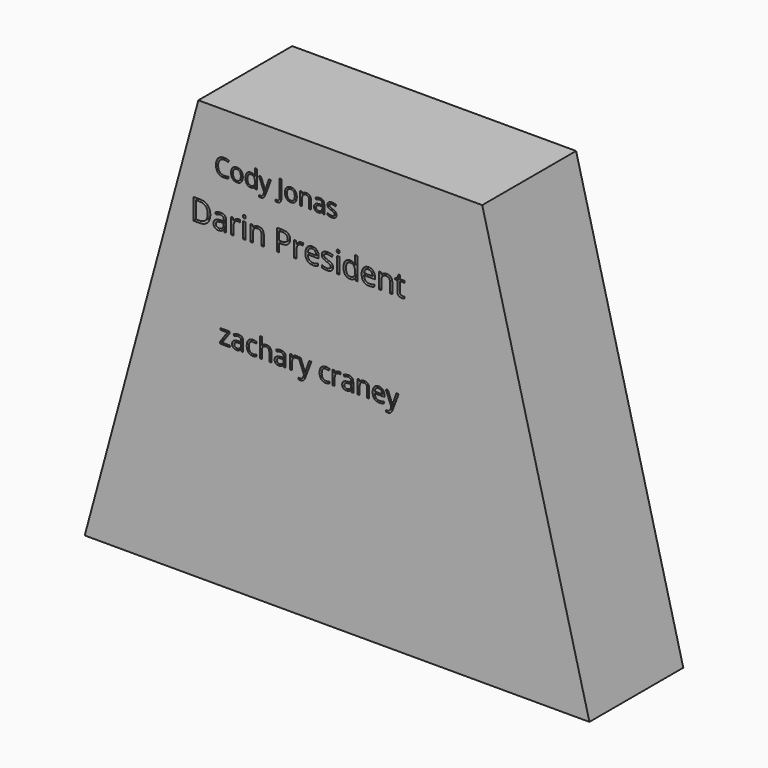
from build123d import *

# Parameters (mm, degrees)
F0_W     = 0.5186502458
F0_H     = 3.4226918918
F1_DEPTH = 25.4


with BuildPart() as f1:
    # F0 (on Front) → F1 (new body)
    with BuildSketch(Plane.XZ):
        Polygon((31.2002788918, 50.6538189948), (-30.2573496559, 50.6538189948), (-54.8576662068, -40.2928031981), (54.4047640278, -40.2928031981), align=None)
        Polygon((-23.4334472811, 6.1464119442), (-23.4334472811, 5.7940250263), (-25.606354207, 5.7940250263), (-25.606354207, 6.1026914829), (-23.9720833641, 8.4364897064), (-25.5049227368, 8.4364897064), (-25.5049227368, 8.7888766243), (-23.4745445147, 8.7888766243), (-23.4745445147, 8.4364897064), (-25.0869551269, 6.1464119442), align=None, mode=Mode.SUBTRACT)
        with BuildLine():
            Line((-20.5531432916, 5.7940250263), (-20.8897908435, 5.7940250263))
            Line((-20.8897908435, 5.7940250263), (-20.9798549937, 6.2207367284))
            Line((-20.9798549937, 6.2207367284), (-21.0017152244, 6.2207367284))
            add(Edge.make_bspline(
                [(-21.0017152244, 6.2207367284), (-21.2255639862, 5.9391769577), (-21.4481011341, 5.8390571014)],
                knots=[0, 0, 0, 1, 1, 1], degree=2))
            add(Edge.make_bspline(
                [(-21.4481011341, 5.8390571014), (-21.6706382821, 5.738937245), (-22.0046626063, 5.738937245)],
                knots=[0, 0, 0, 1, 1, 1], degree=2))
            add(Edge.make_bspline(
                [(-22.0046626063, 5.738937245), (-22.4497369022, 5.738937245), (-22.7024411684, 5.9689068714)],
                knots=[0, 0, 0, 1, 1, 1], degree=2))
            add(Edge.make_bspline(
                [(-22.7024411684, 5.9689068714), (-22.9551454346, 6.1988764978), (-22.9551454346, 6.622090563)],
                knots=[0, 0, 0, 1, 1, 1], degree=2))
            add(Edge.make_bspline(
                [(-22.9551454346, 6.622090563), (-22.9551454346, 7.5288529301), (-21.5045005292, 7.5725733914)],
                knots=[0, 0, 0, 1, 1, 1], degree=2))
            Line((-21.5045005292, 7.5725733914), (-20.996468769, 7.5891871667))
            Line((-20.996468769, 7.5891871667), (-20.996468769, 7.7754363317))
            add(Edge.make_bspline(
                [(-20.996468769, 7.7754363317), (-20.996468769, 8.1278232497), (-21.1477415651, 8.295709821)],
                knots=[0, 0, 0, 1, 1, 1], degree=2))
            add(Edge.make_bspline(
                [(-21.1477415651, 8.295709821), (-21.2990143611, 8.4635963924), (-21.6330386853, 8.4635963924)],
                knots=[0, 0, 0, 1, 1, 1], degree=2))
            add(Edge.make_bspline(
                [(-21.6330386853, 8.4635963924), (-22.007285834, 8.4635963924), (-22.4794668158, 8.2345011752)],
                knots=[0, 0, 0, 1, 1, 1], degree=2))
            Line((-22.4794668158, 8.2345011752), (-22.619372292, 8.5816416378))
            add(Edge.make_bspline(
                [(-22.619372292, 8.5816416378), (-22.3981467578, 8.7014357018), (-22.1345123763, 8.7696396214)],
                knots=[0, 0, 0, 1, 1, 1], degree=2))
            add(Edge.make_bspline(
                [(-22.1345123763, 8.7696396214), (-21.8708779947, 8.837843541), (-21.6050575901, 8.837843541)],
                knots=[0, 0, 0, 1, 1, 1], degree=2))
            add(Edge.make_bspline(
                [(-21.6050575901, 8.837843541), (-21.069919144, 8.837843541), (-20.8115312178, 8.6004414362)],
                knots=[0, 0, 0, 1, 1, 1], degree=2))
            add(Edge.make_bspline(
                [(-20.8115312178, 8.6004414362), (-20.5531432916, 8.3630393314), (-20.5531432916, 7.838393796)],
                knots=[0, 0, 0, 1, 1, 1], degree=2))
            Line((-20.5531432916, 7.838393796), (-20.5531432916, 5.7940250263))
        make_face(mode=Mode.SUBTRACT)
        with BuildLine():
            add(Edge.make_bspline(
                [(-17.6658440283, 5.8954564964), (-17.9657663927, 5.738937245), (-18.4222080085, 5.738937245)],
                knots=[0, 0, 0, 1, 1, 1], degree=2))
            add(Edge.make_bspline(
                [(-18.4222080085, 5.738937245), (-19.0727684724, 5.738937245), (-19.4295274365, 6.1394166704)],
                knots=[0, 0, 0, 1, 1, 1], degree=2))
            add(Edge.make_bspline(
                [(-19.4295274365, 6.1394166704), (-19.7862864006, 6.5398960958), (-19.7862864006, 7.272651027)],
                knots=[0, 0, 0, 1, 1, 1], degree=2))
            add(Edge.make_bspline(
                [(-19.7862864006, 7.272651027), (-19.7862864006, 8.0237685518), (-19.4238437766, 8.4338664787)],
                knots=[0, 0, 0, 1, 1, 1], degree=2))
            add(Edge.make_bspline(
                [(-19.4238437766, 8.4338664787), (-19.0614011525, 8.8439644056), (-18.3924780948, 8.8439644056)],
                knots=[0, 0, 0, 1, 1, 1], degree=2))
            add(Edge.make_bspline(
                [(-18.3924780948, 8.8439644056), (-18.1764990161, 8.8439644056), (-17.9605199373, 8.797183512)],
                knots=[0, 0, 0, 1, 1, 1], degree=2))
            add(Edge.make_bspline(
                [(-17.9605199373, 8.797183512), (-17.7445408586, 8.7504026184), (-17.622123567, 8.6874451542)],
                knots=[0, 0, 0, 1, 1, 1], degree=2))
            Line((-17.622123567, 8.6874451542), (-17.7611546339, 8.3027050948))
            add(Edge.make_bspline(
                [(-17.7611546339, 8.3027050948), (-17.9115530207, 8.3630393314), (-18.0890580935, 8.4023877466)],
                knots=[0, 0, 0, 1, 1, 1], degree=2))
            add(Edge.make_bspline(
                [(-18.0890580935, 8.4023877466), (-18.2665631663, 8.4417361617), (-18.4029710055, 8.4417361617)],
                knots=[0, 0, 0, 1, 1, 1], degree=2))
            add(Edge.make_bspline(
                [(-18.4029710055, 8.4417361617), (-19.3158542372, 8.4417361617), (-19.3158542372, 7.2778974823)],
                knots=[0, 0, 0, 1, 1, 1], degree=2))
            add(Edge.make_bspline(
                [(-19.3158542372, 7.2778974823), (-19.3158542372, 6.7261452609), (-19.0933170892, 6.4310321472)],
                knots=[0, 0, 0, 1, 1, 1], degree=2))
            add(Edge.make_bspline(
                [(-19.0933170892, 6.4310321472), (-18.8707799413, 6.1359190335), (-18.4335753284, 6.1359190335)],
                knots=[0, 0, 0, 1, 1, 1], degree=2))
            add(Edge.make_bspline(
                [(-18.4335753284, 6.1359190335), (-18.0593281798, 6.1359190335), (-17.6658440283, 6.296810331)],
                knots=[0, 0, 0, 1, 1, 1], degree=2))
            Line((-17.6658440283, 6.296810331), (-17.6658440283, 5.8954564964))
        make_face(mode=Mode.SUBTRACT)
        with BuildLine():
            Line((-14.4515157145, 5.7940250263), (-14.9053341027, 5.7940250263))
            Line((-14.9053341027, 5.7940250263), (-14.9053341027, 7.7317158705))
            add(Edge.make_bspline(
                [(-14.9053341027, 7.7317158705), (-14.9053341027, 8.0972189268), (-15.0719090602, 8.2777844319)],
                knots=[0, 0, 0, 1, 1, 1], degree=2))
            add(Edge.make_bspline(
                [(-15.0719090602, 8.2777844319), (-15.2384840177, 8.458349937), (-15.5943685725, 8.458349937)],
                knots=[0, 0, 0, 1, 1, 1], degree=2))
            add(Edge.make_bspline(
                [(-15.5943685725, 8.458349937), (-16.0665495544, 8.458349937), (-16.283840247, 8.2012736247)],
                knots=[0, 0, 0, 1, 1, 1], degree=2))
            add(Edge.make_bspline(
                [(-16.283840247, 8.2012736247), (-16.5011309396, 7.9441973123), (-16.5011309396, 7.3600919495)],
                knots=[0, 0, 0, 1, 1, 1], degree=2))
            Line((-16.5011309396, 7.3600919495), (-16.5011309396, 5.7940250263))
            Line((-16.5011309396, 5.7940250263), (-16.9549493278, 5.7940250263))
            Line((-16.9549493278, 5.7940250263), (-16.9549493278, 10.0462770909))
            Line((-16.9549493278, 10.0462770909), (-16.5011309396, 10.0462770909))
            Line((-16.5011309396, 10.0462770909), (-16.5011309396, 8.7591467107))
            add(Edge.make_bspline(
                [(-16.5011309396, 8.7591467107), (-16.5011309396, 8.5265538566), (-16.5229911703, 8.3735322421)],
                knots=[0, 0, 0, 1, 1, 1], degree=2))
            Line((-16.5229911703, 8.3735322421), (-16.4958844843, 8.3735322421))
            add(Edge.make_bspline(
                [(-16.4958844843, 8.3735322421), (-16.3620998727, 8.5895113209), (-16.1146420618, 8.7136774309)],
                knots=[0, 0, 0, 1, 1, 1], degree=2))
            add(Edge.make_bspline(
                [(-16.1146420618, 8.7136774309), (-15.867184251, 8.837843541), (-15.5506481113, 8.837843541)],
                knots=[0, 0, 0, 1, 1, 1], degree=2))
            add(Edge.make_bspline(
                [(-15.5506481113, 8.837843541), (-15.0015191175, 8.837843541), (-14.726517416, 8.5768323871)],
                knots=[0, 0, 0, 1, 1, 1], degree=2))
            add(Edge.make_bspline(
                [(-14.726517416, 8.5768323871), (-14.4515157145, 8.3158212332), (-14.4515157145, 7.7474552365)],
                knots=[0, 0, 0, 1, 1, 1], degree=2))
            Line((-14.4515157145, 7.7474552365), (-14.4515157145, 5.7940250263))
        make_face(mode=Mode.SUBTRACT)
        with BuildLine():
            Line((-11.3421165079, 5.7940250263), (-11.6787640598, 5.7940250263))
            Line((-11.6787640598, 5.7940250263), (-11.76882821, 6.2207367284))
            Line((-11.76882821, 6.2207367284), (-11.7906884407, 6.2207367284))
            add(Edge.make_bspline(
                [(-11.7906884407, 6.2207367284), (-12.0145372025, 5.9391769577), (-12.2370743504, 5.8390571014)],
                knots=[0, 0, 0, 1, 1, 1], degree=2))
            add(Edge.make_bspline(
                [(-12.2370743504, 5.8390571014), (-12.4596114983, 5.738937245), (-12.7936358226, 5.738937245)],
                knots=[0, 0, 0, 1, 1, 1], degree=2))
            add(Edge.make_bspline(
                [(-12.7936358226, 5.738937245), (-13.2387101185, 5.738937245), (-13.4914143847, 5.9689068714)],
                knots=[0, 0, 0, 1, 1, 1], degree=2))
            add(Edge.make_bspline(
                [(-13.4914143847, 5.9689068714), (-13.7441186509, 6.1988764978), (-13.7441186509, 6.622090563)],
                knots=[0, 0, 0, 1, 1, 1], degree=2))
            add(Edge.make_bspline(
                [(-13.7441186509, 6.622090563), (-13.7441186509, 7.5288529301), (-12.2934737455, 7.5725733914)],
                knots=[0, 0, 0, 1, 1, 1], degree=2))
            Line((-12.2934737455, 7.5725733914), (-11.7854419853, 7.5891871667))
            Line((-11.7854419853, 7.5891871667), (-11.7854419853, 7.7754363317))
            add(Edge.make_bspline(
                [(-11.7854419853, 7.7754363317), (-11.7854419853, 8.1278232497), (-11.9367147814, 8.295709821)],
                knots=[0, 0, 0, 1, 1, 1], degree=2))
            add(Edge.make_bspline(
                [(-11.9367147814, 8.295709821), (-12.0879875774, 8.4635963924), (-12.4220119016, 8.4635963924)],
                knots=[0, 0, 0, 1, 1, 1], degree=2))
            add(Edge.make_bspline(
                [(-12.4220119016, 8.4635963924), (-12.7962590502, 8.4635963924), (-13.2684400321, 8.2345011752)],
                knots=[0, 0, 0, 1, 1, 1], degree=2))
            Line((-13.2684400321, 8.2345011752), (-13.4083455082, 8.5816416378))
            add(Edge.make_bspline(
                [(-13.4083455082, 8.5816416378), (-13.1871199741, 8.7014357018), (-12.9234855926, 8.7696396214)],
                knots=[0, 0, 0, 1, 1, 1], degree=2))
            add(Edge.make_bspline(
                [(-12.9234855926, 8.7696396214), (-12.659851211, 8.837843541), (-12.3940308064, 8.837843541)],
                knots=[0, 0, 0, 1, 1, 1], degree=2))
            add(Edge.make_bspline(
                [(-12.3940308064, 8.837843541), (-11.8588923603, 8.837843541), (-11.6005044341, 8.6004414362)],
                knots=[0, 0, 0, 1, 1, 1], degree=2))
            add(Edge.make_bspline(
                [(-11.6005044341, 8.6004414362), (-11.3421165079, 8.3630393314), (-11.3421165079, 7.838393796)],
                knots=[0, 0, 0, 1, 1, 1], degree=2))
            Line((-11.3421165079, 7.838393796), (-11.3421165079, 5.7940250263))
        make_face(mode=Mode.SUBTRACT)
        with BuildLine():
            add(Edge.make_bspline(
                [(-9.5583216874, 8.6852591311), (-9.3231056057, 8.8439644056), (-9.041545835, 8.8439644056)],
                knots=[0, 0, 0, 1, 1, 1], degree=2))
            add(Edge.make_bspline(
                [(-9.041545835, 8.8439644056), (-8.8421805315, 8.8439644056), (-8.6839124617, 8.810736855)],
                knots=[0, 0, 0, 1, 1, 1], degree=2))
            Line((-8.6839124617, 8.810736855), (-8.7468699259, 8.3901460174))
            add(Edge.make_bspline(
                [(-8.7468699259, 8.3901460174), (-8.9322446818, 8.431243251), (-9.0747733856, 8.431243251)],
                knots=[0, 0, 0, 1, 1, 1], degree=2))
            add(Edge.make_bspline(
                [(-9.0747733856, 8.431243251), (-9.4385276235, 8.431243251), (-9.6964783451, 8.1361301373)],
                knots=[0, 0, 0, 1, 1, 1], degree=2))
            add(Edge.make_bspline(
                [(-9.6964783451, 8.1361301373), (-9.9544290667, 7.8410170237), (-9.9544290667, 7.4011891831)],
                knots=[0, 0, 0, 1, 1, 1], degree=2))
            Line((-9.9544290667, 7.4011891831), (-9.9544290667, 5.7940250263))
            Line((-9.9544290667, 5.7940250263), (-10.4082474548, 5.7940250263))
            Line((-10.4082474548, 5.7940250263), (-10.4082474548, 8.7888766243))
            Line((-10.4082474548, 8.7888766243), (-10.0340003062, 8.7888766243))
            Line((-10.0340003062, 8.7888766243), (-9.9815357527, 8.2345011752))
            Line((-9.9815357527, 8.2345011752), (-9.959675522, 8.2345011752))
            add(Edge.make_bspline(
                [(-9.959675522, 8.2345011752), (-9.7935377691, 8.5265538566), (-9.5583216874, 8.6852591311)],
                knots=[0, 0, 0, 1, 1, 1], degree=2))
        make_face(mode=Mode.SUBTRACT)
        with BuildLine():
            Line((-7.3906612169, 5.777411251), (-8.5990947668, 8.7888766243))
            Line((-8.5990947668, 8.7888766243), (-8.1120488281, 8.7888766243))
            Line((-8.1120488281, 8.7888766243), (-7.4562419088, 7.0811554065))
            add(Edge.make_bspline(
                [(-7.4562419088, 7.0811554065), (-7.2411372393, 6.4961756345), (-7.1886726857, 6.2364760945)],
                knots=[0, 0, 0, 1, 1, 1], degree=2))
            Line((-7.1886726857, 6.2364760945), (-7.1668124551, 6.2364760945))
            add(Edge.make_bspline(
                [(-7.1668124551, 6.2364760945), (-7.131836086, 6.3763815706), (-7.0181628867, 6.7139035317)],
                knots=[0, 0, 0, 1, 1, 1], degree=2))
            add(Edge.make_bspline(
                [(-7.0181628867, 6.7139035317), (-6.9044896874, 7.0514254928), (-6.2757894541, 8.7888766243)],
                knots=[0, 0, 0, 1, 1, 1], degree=2))
            Line((-6.2757894541, 8.7888766243), (-5.7896179246, 8.7888766243))
            Line((-5.7896179246, 8.7888766243), (-7.0767483048, 5.378680644))
            add(Edge.make_bspline(
                [(-7.0767483048, 5.378680644), (-7.2682439253, 4.8732721116), (-7.5235714192, 4.6612278743)],
                knots=[0, 0, 0, 1, 1, 1], degree=2))
            add(Edge.make_bspline(
                [(-7.5235714192, 4.6612278743), (-7.7788989131, 4.4491836371), (-8.150522834, 4.4491836371)],
                knots=[0, 0, 0, 1, 1, 1], degree=2))
            add(Edge.make_bspline(
                [(-8.150522834, 4.4491836371), (-8.3586322297, 4.4491836371), (-8.5606207609, 4.4964017353)],
                knots=[0, 0, 0, 1, 1, 1], degree=2))
            Line((-8.5606207609, 4.4964017353), (-8.5606207609, 4.859281564))
            add(Edge.make_bspline(
                [(-8.5606207609, 4.859281564), (-8.410222374, 4.8269284226), (-8.2248476182, 4.8269284226)],
                knots=[0, 0, 0, 1, 1, 1], degree=2))
            add(Edge.make_bspline(
                [(-8.2248476182, 4.8269284226), (-7.7570386824, 4.8269284226), (-7.557673379, 5.351573958)],
                knots=[0, 0, 0, 1, 1, 1], degree=2))
            Line((-7.557673379, 5.351573958), (-7.3906612169, 5.777411251))
        make_face(mode=Mode.SUBTRACT)
        with BuildLine():
            add(Edge.make_bspline(
                [(-1.8958736424, 5.8954564964), (-2.1957960069, 5.738937245), (-2.6522376227, 5.738937245)],
                knots=[0, 0, 0, 1, 1, 1], degree=2))
            add(Edge.make_bspline(
                [(-2.6522376227, 5.738937245), (-3.3027980866, 5.738937245), (-3.6595570507, 6.1394166704)],
                knots=[0, 0, 0, 1, 1, 1], degree=2))
            add(Edge.make_bspline(
                [(-3.6595570507, 6.1394166704), (-4.0163160148, 6.5398960958), (-4.0163160148, 7.272651027)],
                knots=[0, 0, 0, 1, 1, 1], degree=2))
            add(Edge.make_bspline(
                [(-4.0163160148, 7.272651027), (-4.0163160148, 8.0237685518), (-3.6538733908, 8.4338664787)],
                knots=[0, 0, 0, 1, 1, 1], degree=2))
            add(Edge.make_bspline(
                [(-3.6538733908, 8.4338664787), (-3.2914307667, 8.8439644056), (-2.622507709, 8.8439644056)],
                knots=[0, 0, 0, 1, 1, 1], degree=2))
            add(Edge.make_bspline(
                [(-2.622507709, 8.8439644056), (-2.4065286303, 8.8439644056), (-2.1905495515, 8.797183512)],
                knots=[0, 0, 0, 1, 1, 1], degree=2))
            add(Edge.make_bspline(
                [(-2.1905495515, 8.797183512), (-1.9745704728, 8.7504026184), (-1.8521531812, 8.6874451542)],
                knots=[0, 0, 0, 1, 1, 1], degree=2))
            Line((-1.8521531812, 8.6874451542), (-1.9911842481, 8.3027050948))
            add(Edge.make_bspline(
                [(-1.9911842481, 8.3027050948), (-2.1415826349, 8.3630393314), (-2.3190877077, 8.4023877466)],
                knots=[0, 0, 0, 1, 1, 1], degree=2))
            add(Edge.make_bspline(
                [(-2.3190877077, 8.4023877466), (-2.4965927805, 8.4417361617), (-2.6330006197, 8.4417361617)],
                knots=[0, 0, 0, 1, 1, 1], degree=2))
            add(Edge.make_bspline(
                [(-2.6330006197, 8.4417361617), (-3.5458838514, 8.4417361617), (-3.5458838514, 7.2778974823)],
                knots=[0, 0, 0, 1, 1, 1], degree=2))
            add(Edge.make_bspline(
                [(-3.5458838514, 7.2778974823), (-3.5458838514, 6.7261452609), (-3.3233467034, 6.4310321472)],
                knots=[0, 0, 0, 1, 1, 1], degree=2))
            add(Edge.make_bspline(
                [(-3.3233467034, 6.4310321472), (-3.1008095555, 6.1359190335), (-2.6636049426, 6.1359190335)],
                knots=[0, 0, 0, 1, 1, 1], degree=2))
            add(Edge.make_bspline(
                [(-2.6636049426, 6.1359190335), (-2.289357794, 6.1359190335), (-1.8958736424, 6.296810331)],
                knots=[0, 0, 0, 1, 1, 1], degree=2))
            Line((-1.8958736424, 6.296810331), (-1.8958736424, 5.8954564964))
        make_face(mode=Mode.SUBTRACT)
        with BuildLine():
            add(Edge.make_bspline(
                [(-0.3350531745, 8.6852591311), (-0.0998370928, 8.8439644056), (0.1817226779, 8.8439644056)],
                knots=[0, 0, 0, 1, 1, 1], degree=2))
            add(Edge.make_bspline(
                [(0.1817226779, 8.8439644056), (0.3810879813, 8.8439644056), (0.5393560512, 8.810736855)],
                knots=[0, 0, 0, 1, 1, 1], degree=2))
            Line((0.5393560512, 8.810736855), (0.4763985869, 8.3901460174))
            add(Edge.make_bspline(
                [(0.4763985869, 8.3901460174), (0.2910238311, 8.431243251), (0.1484951273, 8.431243251)],
                knots=[0, 0, 0, 1, 1, 1], degree=2))
            add(Edge.make_bspline(
                [(0.1484951273, 8.431243251), (-0.2152591106, 8.431243251), (-0.4732098322, 8.1361301373)],
                knots=[0, 0, 0, 1, 1, 1], degree=2))
            add(Edge.make_bspline(
                [(-0.4732098322, 8.1361301373), (-0.7311605538, 7.8410170237), (-0.7311605538, 7.4011891831)],
                knots=[0, 0, 0, 1, 1, 1], degree=2))
            Line((-0.7311605538, 7.4011891831), (-0.7311605538, 5.7940250263))
            Line((-0.7311605538, 5.7940250263), (-1.1849789419, 5.7940250263))
            Line((-1.1849789419, 5.7940250263), (-1.1849789419, 8.7888766243))
            Line((-1.1849789419, 8.7888766243), (-0.8107317933, 8.7888766243))
            Line((-0.8107317933, 8.7888766243), (-0.7582672398, 8.2345011752))
            Line((-0.7582672398, 8.2345011752), (-0.7364070091, 8.2345011752))
            add(Edge.make_bspline(
                [(-0.7364070091, 8.2345011752), (-0.5702692563, 8.5265538566), (-0.3350531745, 8.6852591311)],
                knots=[0, 0, 0, 1, 1, 1], degree=2))
        make_face(mode=Mode.SUBTRACT)
        with BuildLine():
            add(Edge.make_bspline(
                [(-28.2644235037, 31.3173672415), (-27.6743214417, 30.7272651795), (-27.6743214417, 29.6679795138)],
                knots=[0, 0, 0, 1, 1, 1], degree=2))
            add(Edge.make_bspline(
                [(-27.6743214417, 29.6679795138), (-27.6743214417, 28.5377416949), (-28.287907667, 27.9396450242)],
                knots=[0, 0, 0, 1, 1, 1], degree=2))
            add(Edge.make_bspline(
                [(-28.287907667, 27.9396450242), (-28.9014938923, 27.3415483534), (-30.0537168854, 27.3415483534)],
                knots=[0, 0, 0, 1, 1, 1], degree=2))
            Line((-30.0537168854, 27.3415483534), (-31.3188637277, 27.3415483534))
            Line((-31.3188637277, 27.3415483534), (-31.3188637277, 31.9074693034))
            Line((-31.3188637277, 31.9074693034), (-29.919807188, 31.9074693034))
            add(Edge.make_bspline(
                [(-29.919807188, 31.9074693034), (-28.8545255656, 31.9074693034), (-28.2644235037, 31.3173672415)],
                knots=[0, 0, 0, 1, 1, 1], degree=2))
        make_face(mode=Mode.SUBTRACT)
        with BuildLine():
            Line((-24.2446342672, 27.3415483534), (-24.6293748157, 27.3415483534))
            Line((-24.6293748157, 27.3415483534), (-24.7323054039, 27.8292194901))
            Line((-24.7323054039, 27.8292194901), (-24.7572885564, 27.8292194901))
            add(Edge.make_bspline(
                [(-24.7572885564, 27.8292194901), (-25.013116038, 27.507436486), (-25.2674445304, 27.3930136476)],
                knots=[0, 0, 0, 1, 1, 1], degree=2))
            add(Edge.make_bspline(
                [(-25.2674445304, 27.3930136476), (-25.5217730228, 27.2785908091), (-25.9035155929, 27.2785908091)],
                knots=[0, 0, 0, 1, 1, 1], degree=2))
            add(Edge.make_bspline(
                [(-25.9035155929, 27.2785908091), (-26.4121725777, 27.2785908091), (-26.7009778205, 27.5414135734)],
                knots=[0, 0, 0, 1, 1, 1], degree=2))
            add(Edge.make_bspline(
                [(-26.7009778205, 27.5414135734), (-26.9897830634, 27.8042363376), (-26.9897830634, 28.2879101699)],
                knots=[0, 0, 0, 1, 1, 1], degree=2))
            add(Edge.make_bspline(
                [(-26.9897830634, 28.2879101699), (-26.9897830634, 29.3242113354), (-25.3319010638, 29.3741776404)],
                knots=[0, 0, 0, 1, 1, 1], degree=2))
            Line((-25.3319010638, 29.3741776404), (-24.7512925998, 29.3931648363))
            Line((-24.7512925998, 29.3931648363), (-24.7512925998, 29.6060212956))
            add(Edge.make_bspline(
                [(-24.7512925998, 29.6060212956), (-24.7512925998, 30.0087497138), (-24.9241760151, 30.200620325)],
                knots=[0, 0, 0, 1, 1, 1], degree=2))
            add(Edge.make_bspline(
                [(-24.9241760151, 30.200620325), (-25.0970594304, 30.3924909361), (-25.4788020005, 30.3924909361)],
                knots=[0, 0, 0, 1, 1, 1], degree=2))
            add(Edge.make_bspline(
                [(-25.4788020005, 30.3924909361), (-25.9065135712, 30.3924909361), (-26.4461496651, 30.130667498)],
                knots=[0, 0, 0, 1, 1, 1], degree=2))
            Line((-26.4461496651, 30.130667498), (-26.6060418411, 30.5273999596))
            add(Edge.make_bspline(
                [(-26.6060418411, 30.5273999596), (-26.3532123378, 30.6643076353), (-26.0519155187, 30.742255071)],
                knots=[0, 0, 0, 1, 1, 1], degree=2))
            add(Edge.make_bspline(
                [(-26.0519155187, 30.742255071), (-25.7506186996, 30.8202025068), (-25.4468235653, 30.8202025068)],
                knots=[0, 0, 0, 1, 1, 1], degree=2))
            add(Edge.make_bspline(
                [(-25.4468235653, 30.8202025068), (-24.8352359922, 30.8202025068), (-24.5399351297, 30.5488854707)],
                knots=[0, 0, 0, 1, 1, 1], degree=2))
            add(Edge.make_bspline(
                [(-24.5399351297, 30.5488854707), (-24.2446342672, 30.2775684346), (-24.2446342672, 29.6779727748)],
                knots=[0, 0, 0, 1, 1, 1], degree=2))
            Line((-24.2446342672, 29.6779727748), (-24.2446342672, 27.3415483534))
        make_face(mode=Mode.SUBTRACT)
        with BuildLine():
            add(Edge.make_bspline(
                [(-22.2060090236, 30.6458201024), (-21.9371903028, 30.8271977895), (-21.6154072987, 30.8271977895)],
                knots=[0, 0, 0, 1, 1, 1], degree=2))
            add(Edge.make_bspline(
                [(-21.6154072987, 30.8271977895), (-21.3875609479, 30.8271977895), (-21.2066829239, 30.7892233977)],
                knots=[0, 0, 0, 1, 1, 1], degree=2))
            Line((-21.2066829239, 30.7892233977), (-21.278634403, 30.3085475437))
            add(Edge.make_bspline(
                [(-21.278634403, 30.3085475437), (-21.4904915362, 30.3555158704), (-21.6533816905, 30.3555158704)],
                knots=[0, 0, 0, 1, 1, 1], degree=2))
            add(Edge.make_bspline(
                [(-21.6533816905, 30.3555158704), (-22.069101348, 30.3555158704), (-22.3639025474, 30.0182433117)],
                knots=[0, 0, 0, 1, 1, 1], degree=2))
            add(Edge.make_bspline(
                [(-22.3639025474, 30.0182433117), (-22.6587037469, 29.6809707531), (-22.6587037469, 29.1783097249)],
                knots=[0, 0, 0, 1, 1, 1], degree=2))
            Line((-22.6587037469, 29.1783097249), (-22.6587037469, 27.3415483534))
            Line((-22.6587037469, 27.3415483534), (-23.1773539927, 27.3415483534))
            Line((-23.1773539927, 27.3415483534), (-23.1773539927, 30.7642402452))
            Line((-23.1773539927, 30.7642402452), (-22.7496424219, 30.7642402452))
            Line((-22.7496424219, 30.7642402452), (-22.6896828559, 30.130667498))
            Line((-22.6896828559, 30.130667498), (-22.6646997035, 30.130667498))
            add(Edge.make_bspline(
                [(-22.6646997035, 30.130667498), (-22.4748277445, 30.4644424153), (-22.2060090236, 30.6458201024)],
                knots=[0, 0, 0, 1, 1, 1], degree=2))
        make_face(mode=Mode.SUBTRACT)
        with Locations((-20.306789771, 29.0528942993)):
            Rectangle(F0_W, F0_H, mode=Mode.SUBTRACT)
        with BuildLine():
            Line((-16.0871353146, 27.3415483534), (-16.6057855604, 27.3415483534))
            Line((-16.6057855604, 27.3415483534), (-16.6057855604, 29.5560549906))
            add(Edge.make_bspline(
                [(-16.6057855604, 29.5560549906), (-16.6057855604, 29.9737733003), (-16.7961571824, 30.1801341399)],
                knots=[0, 0, 0, 1, 1, 1], degree=2))
            add(Edge.make_bspline(
                [(-16.7961571824, 30.1801341399), (-16.9865288044, 30.3864949795), (-17.393254527, 30.3864949795)],
                knots=[0, 0, 0, 1, 1, 1], degree=2))
            add(Edge.make_bspline(
                [(-17.393254527, 30.3864949795), (-17.9298926426, 30.3864949795), (-18.1797241676, 30.0961907475)],
                knots=[0, 0, 0, 1, 1, 1], degree=2))
            add(Edge.make_bspline(
                [(-18.1797241676, 30.0961907475), (-18.4295556925, 29.8058865155), (-18.4295556925, 29.1373373548)],
                knots=[0, 0, 0, 1, 1, 1], degree=2))
            Line((-18.4295556925, 29.1373373548), (-18.4295556925, 27.3415483534))
            Line((-18.4295556925, 27.3415483534), (-18.9482059383, 27.3415483534))
            Line((-18.9482059383, 27.3415483534), (-18.9482059383, 30.7642402452))
            Line((-18.9482059383, 30.7642402452), (-18.5264903242, 30.7642402452))
            Line((-18.5264903242, 30.7642402452), (-18.4425469318, 30.2955563044))
            Line((-18.4425469318, 30.2955563044), (-18.4175637793, 30.2955563044))
            add(Edge.make_bspline(
                [(-18.4175637793, 30.2955563044), (-18.2576716034, 30.5483858077), (-17.9703653497, 30.6877917986)],
                knots=[0, 0, 0, 1, 1, 1], degree=2))
            add(Edge.make_bspline(
                [(-17.9703653497, 30.6877917986), (-17.683059096, 30.8271977895), (-17.3302969827, 30.8271977895)],
                knots=[0, 0, 0, 1, 1, 1], degree=2))
            add(Edge.make_bspline(
                [(-17.3302969827, 30.8271977895), (-16.711714127, 30.8271977895), (-16.3994247208, 30.5288989487)],
                knots=[0, 0, 0, 1, 1, 1], degree=2))
            add(Edge.make_bspline(
                [(-16.3994247208, 30.5288989487), (-16.0871353146, 30.2306001079), (-16.0871353146, 29.5740428604)],
                knots=[0, 0, 0, 1, 1, 1], degree=2))
            Line((-16.0871353146, 29.5740428604), (-16.0871353146, 27.3415483534))
        make_face(mode=Mode.SUBTRACT)
        with BuildLine():
            add(Edge.make_bspline(
                [(-20.5226442085, 31.4307907538), (-20.6100852423, 31.5167327984), (-20.6100852423, 31.6916148658)],
                knots=[0, 0, 0, 1, 1, 1], degree=2))
            add(Edge.make_bspline(
                [(-20.6100852423, 31.6916148658), (-20.6100852423, 31.8694949116), (-20.5226442085, 31.9524389779)],
                knots=[0, 0, 0, 1, 1, 1], degree=2))
            add(Edge.make_bspline(
                [(-20.5226442085, 31.9524389779), (-20.4352031748, 32.0353830442), (-20.3032921296, 32.0353830442)],
                knots=[0, 0, 0, 1, 1, 1], degree=2))
            add(Edge.make_bspline(
                [(-20.3032921296, 32.0353830442), (-20.1783763672, 32.0353830442), (-20.0879373551, 31.9509399887)],
                knots=[0, 0, 0, 1, 1, 1], degree=2))
            add(Edge.make_bspline(
                [(-20.0879373551, 31.9509399887), (-19.9974983431, 31.8664969333), (-19.9974983431, 31.6916148658)],
                knots=[0, 0, 0, 1, 1, 1], degree=2))
            add(Edge.make_bspline(
                [(-19.9974983431, 31.6916148658), (-19.9974983431, 31.5167327984), (-20.0879373551, 31.4307907538)],
                knots=[0, 0, 0, 1, 1, 1], degree=2))
            add(Edge.make_bspline(
                [(-20.0879373551, 31.4307907538), (-20.1783763672, 31.3448487092), (-20.3032921296, 31.3448487092)],
                knots=[0, 0, 0, 1, 1, 1], degree=2))
            add(Edge.make_bspline(
                [(-20.3032921296, 31.3448487092), (-20.4352031748, 31.3448487092), (-20.5226442085, 31.4307907538)],
                knots=[0, 0, 0, 1, 1, 1], degree=2))
        make_face(mode=Mode.SUBTRACT)
        with BuildLine():
            add(Edge.make_bspline(
                [(-20.9723246593, 40.1999839859), (-20.6284628156, 39.8114647598), (-20.6284628156, 39.1497235493)],
                knots=[0, 0, 0, 1, 1, 1], degree=2))
            add(Edge.make_bspline(
                [(-20.6284628156, 39.1497235493), (-20.6284628156, 38.4693074334), (-20.9707007545, 38.0872838266)],
                knots=[0, 0, 0, 1, 1, 1], degree=2))
            add(Edge.make_bspline(
                [(-20.9707007545, 38.0872838266), (-21.3129386935, 37.7052602198), (-21.9170312832, 37.7052602198)],
                knots=[0, 0, 0, 1, 1, 1], degree=2))
            add(Edge.make_bspline(
                [(-21.9170312832, 37.7052602198), (-22.2905293898, 37.7052602198), (-22.5795844461, 37.8806419394)],
                knots=[0, 0, 0, 1, 1, 1], degree=2))
            add(Edge.make_bspline(
                [(-22.5795844461, 37.8806419394), (-22.8686395025, 38.056023659), (-23.0261582692, 38.3832404784)],
                knots=[0, 0, 0, 1, 1, 1], degree=2))
            add(Edge.make_bspline(
                [(-23.0261582692, 38.3832404784), (-23.1836770359, 38.7104572979), (-23.1836770359, 39.1497235493)],
                knots=[0, 0, 0, 1, 1, 1], degree=2))
            add(Edge.make_bspline(
                [(-23.1836770359, 39.1497235493), (-23.1836770359, 39.8293277127), (-22.843468978, 40.2089154623)],
                knots=[0, 0, 0, 1, 1, 1], degree=2))
            add(Edge.make_bspline(
                [(-22.843468978, 40.2089154623), (-22.50326092, 40.5885032119), (-21.8991683303, 40.5885032119)],
                knots=[0, 0, 0, 1, 1, 1], degree=2))
            add(Edge.make_bspline(
                [(-21.8991683303, 40.5885032119), (-21.3161865031, 40.5885032119), (-20.9723246593, 40.1999839859)],
                knots=[0, 0, 0, 1, 1, 1], degree=2))
        make_face(mode=Mode.SUBTRACT)
        with BuildLine():
            Line((-16.0246926761, 37.7409861257), (-17.1468109006, 40.5373502104))
            Line((-17.1468109006, 40.5373502104), (-16.6945534107, 40.5373502104))
            Line((-16.6945534107, 40.5373502104), (-16.0855891065, 38.9516071623))
            add(Edge.make_bspline(
                [(-16.0855891065, 38.9516071623), (-15.8858488147, 38.408411003), (-15.8371316704, 38.1672611386)],
                knots=[0, 0, 0, 1, 1, 1], degree=2))
            Line((-15.8371316704, 38.1672611386), (-15.8168328603, 38.1672611386))
            add(Edge.make_bspline(
                [(-15.8168328603, 38.1672611386), (-15.784354764, 38.2971735235), (-15.6788009513, 38.610587152)],
                knots=[0, 0, 0, 1, 1, 1], degree=2))
            add(Edge.make_bspline(
                [(-15.6788009513, 38.610587152), (-15.5732471386, 38.9240007806), (-14.989453359, 40.5373502104)],
                knots=[0, 0, 0, 1, 1, 1], degree=2))
            Line((-14.989453359, 40.5373502104), (-14.5380078215, 40.5373502104))
            Line((-14.5380078215, 40.5373502104), (-15.7332017625, 37.3707358287))
            add(Edge.make_bspline(
                [(-15.7332017625, 37.3707358287), (-15.9110193393, 36.9014273383), (-16.1481094417, 36.70452888)],
                knots=[0, 0, 0, 1, 1, 1], degree=2))
            add(Edge.make_bspline(
                [(-16.1481094417, 36.70452888), (-16.3851995441, 36.5076304216), (-16.7302793165, 36.5076304216)],
                knots=[0, 0, 0, 1, 1, 1], degree=2))
            add(Edge.make_bspline(
                [(-16.7302793165, 36.5076304216), (-16.923523989, 36.5076304216), (-17.1110849947, 36.5514758515)],
                knots=[0, 0, 0, 1, 1, 1], degree=2))
            Line((-17.1110849947, 36.5514758515), (-17.1110849947, 36.8884360998))
            add(Edge.make_bspline(
                [(-17.1110849947, 36.8884360998), (-16.971429181, 36.8583938608), (-16.799295271, 36.8583938608)],
                knots=[0, 0, 0, 1, 1, 1], degree=2))
            add(Edge.make_bspline(
                [(-16.799295271, 36.8583938608), (-16.364900734, 36.8583938608), (-16.1797755855, 37.3455653041)],
                knots=[0, 0, 0, 1, 1, 1], degree=2))
            Line((-16.1797755855, 37.3455653041), (-16.0246926761, 37.7409861257))
        make_face(mode=Mode.SUBTRACT)
        with BuildLine():
            add(Edge.make_bspline(
                [(-12.0988248503, 31.9074693034), (-10.3879785675, 31.9074693034), (-10.3879785675, 30.5773662646)],
                knots=[0, 0, 0, 1, 1, 1], degree=2))
            add(Edge.make_bspline(
                [(-10.3879785675, 30.5773662646), (-10.3879785675, 29.8838339513), (-10.8611594757, 29.510585653)],
                knots=[0, 0, 0, 1, 1, 1], degree=2))
            add(Edge.make_bspline(
                [(-10.8611594757, 29.510585653), (-11.334340384, 29.1373373548), (-12.2147466779, 29.1373373548)],
                knots=[0, 0, 0, 1, 1, 1], degree=2))
            Line((-12.2147466779, 29.1373373548), (-12.7523841196, 29.1373373548))
            Line((-12.7523841196, 29.1373373548), (-12.7523841196, 27.3415483534))
            Line((-12.7523841196, 27.3415483534), (-13.2830262786, 27.3415483534))
            Line((-13.2830262786, 27.3415483534), (-13.2830262786, 31.9074693034))
            Line((-13.2830262786, 31.9074693034), (-12.0988248503, 31.9074693034))
        make_face(mode=Mode.SUBTRACT)
        with BuildLine():
            add(Edge.make_bspline(
                [(-8.5392252828, 30.6458201024), (-8.270406562, 30.8271977895), (-7.9486235578, 30.8271977895)],
                knots=[0, 0, 0, 1, 1, 1], degree=2))
            add(Edge.make_bspline(
                [(-7.9486235578, 30.8271977895), (-7.7207772071, 30.8271977895), (-7.539899183, 30.7892233977)],
                knots=[0, 0, 0, 1, 1, 1], degree=2))
            Line((-7.539899183, 30.7892233977), (-7.6118506622, 30.3085475437))
            add(Edge.make_bspline(
                [(-7.6118506622, 30.3085475437), (-7.8237077954, 30.3555158704), (-7.9865979496, 30.3555158704)],
                knots=[0, 0, 0, 1, 1, 1], degree=2))
            add(Edge.make_bspline(
                [(-7.9865979496, 30.3555158704), (-8.4023176072, 30.3555158704), (-8.6971188066, 30.0182433117)],
                knots=[0, 0, 0, 1, 1, 1], degree=2))
            add(Edge.make_bspline(
                [(-8.6971188066, 30.0182433117), (-8.991920006, 29.6809707531), (-8.991920006, 29.1783097249)],
                knots=[0, 0, 0, 1, 1, 1], degree=2))
            Line((-8.991920006, 29.1783097249), (-8.991920006, 27.3415483534))
            Line((-8.991920006, 27.3415483534), (-9.5105702518, 27.3415483534))
            Line((-9.5105702518, 27.3415483534), (-9.5105702518, 30.7642402452))
            Line((-9.5105702518, 30.7642402452), (-9.0828586811, 30.7642402452))
            Line((-9.0828586811, 30.7642402452), (-9.0228991151, 30.130667498))
            Line((-9.0228991151, 30.130667498), (-8.9979159626, 30.130667498))
            add(Edge.make_bspline(
                [(-8.9979159626, 30.130667498), (-8.8080440037, 30.4644424153), (-8.5392252828, 30.6458201024)],
                knots=[0, 0, 0, 1, 1, 1], degree=2))
        make_face(mode=Mode.SUBTRACT)
        with BuildLine():
            add(Edge.make_bspline(
                [(-4.8617052356, 27.3305557663), (-5.10654013, 27.2785908091), (-5.4533062867, 27.2785908091)],
                knots=[0, 0, 0, 1, 1, 1], degree=2))
            add(Edge.make_bspline(
                [(-5.4533062867, 27.2785908091), (-6.2117947964, 27.2785908091), (-6.6509986173, 27.7412787934)],
                knots=[0, 0, 0, 1, 1, 1], degree=2))
            add(Edge.make_bspline(
                [(-6.6509986173, 27.7412787934), (-7.0902024381, 28.2039667776), (-7.0902024381, 29.0244135055)],
                knots=[0, 0, 0, 1, 1, 1], degree=2))
            add(Edge.make_bspline(
                [(-7.0902024381, 29.0244135055), (-7.0902024381, 29.8528548422), (-6.6824773894, 30.3400263159)],
                knots=[0, 0, 0, 1, 1, 1], degree=2))
            add(Edge.make_bspline(
                [(-6.6824773894, 30.3400263159), (-6.2747523407, 30.8271977895), (-5.587215984, 30.8271977895)],
                knots=[0, 0, 0, 1, 1, 1], degree=2))
            add(Edge.make_bspline(
                [(-5.587215984, 30.8271977895), (-4.9446493019, 30.8271977895), (-4.5699020144, 30.4039831863)],
                knots=[0, 0, 0, 1, 1, 1], degree=2))
            add(Edge.make_bspline(
                [(-4.5699020144, 30.4039831863), (-4.195154727, 29.980768583), (-4.195154727, 29.2872362697)],
                knots=[0, 0, 0, 1, 1, 1], degree=2))
            Line((-4.195154727, 29.2872362697), (-4.195154727, 28.959457309))
            Line((-4.195154727, 28.959457309), (-6.5525649964, 28.959457309))
            add(Edge.make_bspline(
                [(-6.5525649964, 28.959457309), (-6.5365757788, 28.3568636708), (-6.247770536, 28.0445742646)],
                knots=[0, 0, 0, 1, 1, 1], degree=2))
            add(Edge.make_bspline(
                [(-6.247770536, 28.0445742646), (-5.9589652932, 27.7322848585), (-5.4343190908, 27.7322848585)],
                knots=[0, 0, 0, 1, 1, 1], degree=2))
            add(Edge.make_bspline(
                [(-5.4343190908, 27.7322848585), (-4.8816917576, 27.7322848585), (-4.3420556637, 27.9631291875)],
                knots=[0, 0, 0, 1, 1, 1], degree=2))
            Line((-4.3420556637, 27.9631291875), (-4.3420556637, 27.5004412033))
            add(Edge.make_bspline(
                [(-4.3420556637, 27.5004412033), (-4.6168703411, 27.3825207235), (-4.8617052356, 27.3305557663)],
                knots=[0, 0, 0, 1, 1, 1], degree=2))
        make_face(mode=Mode.SUBTRACT)
        with BuildLine():
            add(Edge.make_bspline(
                [(-1.3170955596, 28.8405375031), (-1.1032397742, 28.6156891307), (-1.1032397742, 28.2749189306)],
                knots=[0, 0, 0, 1, 1, 1], degree=2))
            add(Edge.make_bspline(
                [(-1.1032397742, 28.2749189306), (-1.1032397742, 27.7972410549), (-1.4589998658, 27.537915932)],
                knots=[0, 0, 0, 1, 1, 1], degree=2))
            add(Edge.make_bspline(
                [(-1.4589998658, 27.537915932), (-1.8147599573, 27.2785908091), (-2.4583259656, 27.2785908091)],
                knots=[0, 0, 0, 1, 1, 1], degree=2))
            add(Edge.make_bspline(
                [(-2.4583259656, 27.2785908091), (-3.1388670395, 27.2785908091), (-3.5196102835, 27.4944452467)],
                knots=[0, 0, 0, 1, 1, 1], degree=2))
            Line((-3.5196102835, 27.4944452467), (-3.5196102835, 27.9751211007))
            add(Edge.make_bspline(
                [(-3.5196102835, 27.9751211007), (-3.2727767369, 27.8502053382), (-2.9904671137, 27.7787535221)],
                knots=[0, 0, 0, 1, 1, 1], degree=2))
            add(Edge.make_bspline(
                [(-2.9904671137, 27.7787535221), (-2.7081574905, 27.707301706), (-2.4453347263, 27.707301706)],
                knots=[0, 0, 0, 1, 1, 1], degree=2))
            add(Edge.make_bspline(
                [(-2.4453347263, 27.707301706), (-2.0396083297, 27.707301706), (-1.8212555769, 27.8367144359)],
                knots=[0, 0, 0, 1, 1, 1], degree=2))
            add(Edge.make_bspline(
                [(-1.8212555769, 27.8367144359), (-1.6029028241, 27.9661271658), (-1.6029028241, 28.2319479084)],
                knots=[0, 0, 0, 1, 1, 1], degree=2))
            add(Edge.make_bspline(
                [(-1.6029028241, 28.2319479084), (-1.6029028241, 28.4318131283), (-1.7757862394, 28.5737174345)],
                knots=[0, 0, 0, 1, 1, 1], degree=2))
            add(Edge.make_bspline(
                [(-1.7757862394, 28.5737174345), (-1.9486696547, 28.7156217407), (-2.452330009, 28.909491004)],
                knots=[0, 0, 0, 1, 1, 1], degree=2))
            add(Edge.make_bspline(
                [(-2.452330009, 28.909491004), (-2.9300078847, 29.0873710498), (-3.1313720938, 29.2202814211)],
                knots=[0, 0, 0, 1, 1, 1], degree=2))
            add(Edge.make_bspline(
                [(-3.1313720938, 29.2202814211), (-3.3327363029, 29.3531917923), (-3.4311699237, 29.5215782401)],
                knots=[0, 0, 0, 1, 1, 1], degree=2))
            add(Edge.make_bspline(
                [(-3.4311699237, 29.5215782401), (-3.5296035445, 29.689964688), (-3.5296035445, 29.9238069953)],
                knots=[0, 0, 0, 1, 1, 1], degree=2))
            add(Edge.make_bspline(
                [(-3.5296035445, 29.9238069953), (-3.5296035445, 30.3425246311), (-3.1888333445, 30.5848612103)],
                knots=[0, 0, 0, 1, 1, 1], degree=2))
            add(Edge.make_bspline(
                [(-3.1888333445, 30.5848612103), (-2.8480631445, 30.8271977895), (-2.2554627673, 30.8271977895)],
                knots=[0, 0, 0, 1, 1, 1], degree=2))
            add(Edge.make_bspline(
                [(-2.2554627673, 30.8271977895), (-1.7028354341, 30.8271977895), (-1.1741919273, 30.6023494171)],
                knots=[0, 0, 0, 1, 1, 1], degree=2))
            Line((-1.1741919273, 30.6023494171), (-1.3590672558, 30.180633803))
            add(Edge.make_bspline(
                [(-1.3590672558, 30.180633803), (-1.8737201972, 30.3924909361), (-2.292437833, 30.3924909361)],
                knots=[0, 0, 0, 1, 1, 1], degree=2))
            add(Edge.make_bspline(
                [(-2.292437833, 30.3924909361), (-2.6611891638, 30.3924909361), (-2.8485628075, 30.2770687716)],
                knots=[0, 0, 0, 1, 1, 1], degree=2))
            add(Edge.make_bspline(
                [(-2.8485628075, 30.2770687716), (-3.0359364512, 30.1616466071), (-3.0359364512, 29.9587834088)],
                knots=[0, 0, 0, 1, 1, 1], degree=2))
            add(Edge.make_bspline(
                [(-3.0359364512, 29.9587834088), (-3.0359364512, 29.820876407), (-2.9654839612, 29.7244414384)],
                knots=[0, 0, 0, 1, 1, 1], degree=2))
            add(Edge.make_bspline(
                [(-2.9654839612, 29.7244414384), (-2.8950314712, 29.6280064698), (-2.7391365996, 29.540565436)],
                knots=[0, 0, 0, 1, 1, 1], degree=2))
            add(Edge.make_bspline(
                [(-2.7391365996, 29.540565436), (-2.583241728, 29.4531244023), (-2.1395409397, 29.2872362697)],
                knots=[0, 0, 0, 1, 1, 1], degree=2))
            add(Edge.make_bspline(
                [(-2.1395409397, 29.2872362697), (-1.530951345, 29.0653858756), (-1.3170955596, 28.8405375031)],
                knots=[0, 0, 0, 1, 1, 1], degree=2))
        make_face(mode=Mode.SUBTRACT)
        with BuildLine():
            add(Edge.make_bspline(
                [(-12.512998522, 37.0447369379), (-12.7565842437, 36.7796344775), (-13.213713448, 36.7796344775)],
                knots=[0, 0, 0, 1, 1, 1], degree=2))
            add(Edge.make_bspline(
                [(-13.213713448, 36.7796344775), (-13.4516155029, 36.7796344775), (-13.5888354594, 36.8478384795)],
                knots=[0, 0, 0, 1, 1, 1], degree=2))
            Line((-13.5888354594, 36.8478384795), (-13.5888354594, 37.2156529193))
            add(Edge.make_bspline(
                [(-13.5888354594, 37.2156529193), (-13.4085820254, 37.1653118701), (-13.213713448, 37.1653118701)],
                knots=[0, 0, 0, 1, 1, 1], degree=2))
            add(Edge.make_bspline(
                [(-13.213713448, 37.1653118701), (-12.9620082023, 37.1653118701), (-12.831283865, 37.3175529462)],
                knots=[0, 0, 0, 1, 1, 1], degree=2))
            add(Edge.make_bspline(
                [(-12.831283865, 37.3175529462), (-12.7005595277, 37.4697940222), (-12.7005595277, 37.7564132214)],
                knots=[0, 0, 0, 1, 1, 1], degree=2))
            Line((-12.7005595277, 37.7564132214), (-12.7005595277, 41.4662237624))
            Line((-12.7005595277, 41.4662237624), (-12.2694128004, 41.4662237624))
            Line((-12.2694128004, 41.4662237624), (-12.2694128004, 37.7921391272))
            add(Edge.make_bspline(
                [(-12.2694128004, 37.7921391272), (-12.2694128004, 37.3098393983), (-12.512998522, 37.0447369379)],
                knots=[0, 0, 0, 1, 1, 1], degree=2))
        make_face(mode=Mode.SUBTRACT)
        with BuildLine():
            add(Edge.make_bspline(
                [(-9.2923893054, 40.1999839859), (-8.9485274616, 39.8114647598), (-8.9485274616, 39.1497235493)],
                knots=[0, 0, 0, 1, 1, 1], degree=2))
            add(Edge.make_bspline(
                [(-8.9485274616, 39.1497235493), (-8.9485274616, 38.4693074334), (-9.2907654006, 38.0872838266)],
                knots=[0, 0, 0, 1, 1, 1], degree=2))
            add(Edge.make_bspline(
                [(-9.2907654006, 38.0872838266), (-9.6330033395, 37.7052602198), (-10.2370959293, 37.7052602198)],
                knots=[0, 0, 0, 1, 1, 1], degree=2))
            add(Edge.make_bspline(
                [(-10.2370959293, 37.7052602198), (-10.6105940358, 37.7052602198), (-10.8996490922, 37.8806419394)],
                knots=[0, 0, 0, 1, 1, 1], degree=2))
            add(Edge.make_bspline(
                [(-10.8996490922, 37.8806419394), (-11.1887041486, 38.056023659), (-11.3462229153, 38.3832404784)],
                knots=[0, 0, 0, 1, 1, 1], degree=2))
            add(Edge.make_bspline(
                [(-11.3462229153, 38.3832404784), (-11.5037416819, 38.7104572979), (-11.5037416819, 39.1497235493)],
                knots=[0, 0, 0, 1, 1, 1], degree=2))
            add(Edge.make_bspline(
                [(-11.5037416819, 39.1497235493), (-11.5037416819, 39.8293277127), (-11.163533624, 40.2089154623)],
                knots=[0, 0, 0, 1, 1, 1], degree=2))
            add(Edge.make_bspline(
                [(-11.163533624, 40.2089154623), (-10.8233255661, 40.5885032119), (-10.2192329763, 40.5885032119)],
                knots=[0, 0, 0, 1, 1, 1], degree=2))
            add(Edge.make_bspline(
                [(-10.2192329763, 40.5885032119), (-9.6362511492, 40.5885032119), (-9.2923893054, 40.1999839859)],
                knots=[0, 0, 0, 1, 1, 1], degree=2))
        make_face(mode=Mode.SUBTRACT)
        with BuildLine():
            Line((-5.8850310355, 37.7564132214), (-6.306434334, 37.7564132214))
            Line((-6.306434334, 37.7564132214), (-6.306434334, 39.5556997521))
            add(Edge.make_bspline(
                [(-6.306434334, 39.5556997521), (-6.306434334, 39.8950958576), (-6.4611112672, 40.0627640293)],
                knots=[0, 0, 0, 1, 1, 1], degree=2))
            add(Edge.make_bspline(
                [(-6.4611112672, 40.0627640293), (-6.6157882005, 40.2304322011), (-6.9462528295, 40.2304322011)],
                knots=[0, 0, 0, 1, 1, 1], degree=2))
            add(Edge.make_bspline(
                [(-6.9462528295, 40.2304322011), (-7.3822712713, 40.2304322011), (-7.5852593727, 39.9945600273)],
                knots=[0, 0, 0, 1, 1, 1], degree=2))
            add(Edge.make_bspline(
                [(-7.5852593727, 39.9945600273), (-7.7882474741, 39.7586878535), (-7.7882474741, 39.2154916941)],
                knots=[0, 0, 0, 1, 1, 1], degree=2))
            Line((-7.7882474741, 39.2154916941), (-7.7882474741, 37.7564132214))
            Line((-7.7882474741, 37.7564132214), (-8.2096507726, 37.7564132214))
            Line((-8.2096507726, 37.7564132214), (-8.2096507726, 40.5373502104))
            Line((-8.2096507726, 40.5373502104), (-7.8670068574, 40.5373502104))
            Line((-7.8670068574, 40.5373502104), (-7.7988028554, 40.1565445322))
            Line((-7.7988028554, 40.1565445322), (-7.7785040452, 40.1565445322))
            add(Edge.make_bspline(
                [(-7.7785040452, 40.1565445322), (-7.6485916604, 40.3619684908), (-7.4151553438, 40.4752358514)],
                knots=[0, 0, 0, 1, 1, 1], degree=2))
            add(Edge.make_bspline(
                [(-7.4151553438, 40.4752358514), (-7.1817190272, 40.5885032119), (-6.895099828, 40.5885032119)],
                knots=[0, 0, 0, 1, 1, 1], degree=2))
            add(Edge.make_bspline(
                [(-6.895099828, 40.5885032119), (-6.392501289, 40.5885032119), (-6.1387661622, 40.3461354189)],
                knots=[0, 0, 0, 1, 1, 1], degree=2))
            add(Edge.make_bspline(
                [(-6.1387661622, 40.3461354189), (-5.8850310355, 40.1037676258), (-5.8850310355, 39.5703148954)],
                knots=[0, 0, 0, 1, 1, 1], degree=2))
            Line((-5.8850310355, 39.5703148954), (-5.8850310355, 37.7564132214))
        make_face(mode=Mode.SUBTRACT)
        with BuildLine():
            Line((-2.9977282813, 37.7564132214), (-3.3103299575, 37.7564132214))
            Line((-3.3103299575, 37.7564132214), (-3.3939610552, 38.1526459953))
            Line((-3.3939610552, 38.1526459953), (-3.4142598654, 38.1526459953))
            add(Edge.make_bspline(
                [(-3.4142598654, 38.1526459953), (-3.6221196812, 37.8911973207), (-3.8287615684, 37.7982287702)],
                knots=[0, 0, 0, 1, 1, 1], degree=2))
            add(Edge.make_bspline(
                [(-3.8287615684, 37.7982287702), (-4.0354034556, 37.7052602198), (-4.3455692745, 37.7052602198)],
                knots=[0, 0, 0, 1, 1, 1], degree=2))
            add(Edge.make_bspline(
                [(-4.3455692745, 37.7052602198), (-4.758853049, 37.7052602198), (-4.9935072942, 37.9188037025)],
                knots=[0, 0, 0, 1, 1, 1], degree=2))
            add(Edge.make_bspline(
                [(-4.9935072942, 37.9188037025), (-5.2281615394, 38.1323471851), (-5.2281615394, 38.5253321494)],
                knots=[0, 0, 0, 1, 1, 1], degree=2))
            add(Edge.make_bspline(
                [(-5.2281615394, 38.5253321494), (-5.2281615394, 39.367326794), (-3.8811324986, 39.4079244143)],
                knots=[0, 0, 0, 1, 1, 1], degree=2))
            Line((-3.8811324986, 39.4079244143), (-3.4093881509, 39.42335151))
            Line((-3.4093881509, 39.42335151), (-3.4093881509, 39.5962973724))
            add(Edge.make_bspline(
                [(-3.4093881509, 39.5962973724), (-3.4093881509, 39.9235141918), (-3.5498559171, 40.0794090537)],
                knots=[0, 0, 0, 1, 1, 1], degree=2))
            add(Edge.make_bspline(
                [(-3.5498559171, 40.0794090537), (-3.6903236833, 40.2353039155), (-4.0004895022, 40.2353039155)],
                knots=[0, 0, 0, 1, 1, 1], degree=2))
            add(Edge.make_bspline(
                [(-4.0004895022, 40.2353039155), (-4.3480051318, 40.2353039155), (-4.7864594308, 40.0225723853)],
                knots=[0, 0, 0, 1, 1, 1], degree=2))
            Line((-4.7864594308, 40.0225723853), (-4.9163718157, 40.3449174903))
            add(Edge.make_bspline(
                [(-4.9163718157, 40.3449174903), (-4.710947857, 40.4561549698), (-4.4661442068, 40.5194872575)],
                knots=[0, 0, 0, 1, 1, 1], degree=2))
            add(Edge.make_bspline(
                [(-4.4661442068, 40.5194872575), (-4.2213405565, 40.5828195451), (-3.9745070252, 40.5828195451)],
                knots=[0, 0, 0, 1, 1, 1], degree=2))
            add(Edge.make_bspline(
                [(-3.9745070252, 40.5828195451), (-3.477592153, 40.5828195451), (-3.2376602172, 40.362374467)],
                knots=[0, 0, 0, 1, 1, 1], degree=2))
            add(Edge.make_bspline(
                [(-3.2376602172, 40.362374467), (-2.9977282813, 40.1419293889), (-2.9977282813, 39.6547579456)],
                knots=[0, 0, 0, 1, 1, 1], degree=2))
            Line((-2.9977282813, 39.6547579456), (-2.9977282813, 37.7564132214))
        make_face(mode=Mode.SUBTRACT)
        with BuildLine():
            add(Edge.make_bspline(
                [(-0.5107180631, 38.9743418297), (-0.3369602483, 38.7916525384), (-0.3369602483, 38.5147767681)],
                knots=[0, 0, 0, 1, 1, 1], degree=2))
            add(Edge.make_bspline(
                [(-0.3369602483, 38.5147767681), (-0.3369602483, 38.1266635183), (-0.6260153047, 37.9159618691)],
                knots=[0, 0, 0, 1, 1, 1], degree=2))
            add(Edge.make_bspline(
                [(-0.6260153047, 37.9159618691), (-0.9150703611, 37.7052602198), (-1.4379677102, 37.7052602198)],
                knots=[0, 0, 0, 1, 1, 1], degree=2))
            add(Edge.make_bspline(
                [(-1.4379677102, 37.7052602198), (-1.9909072984, 37.7052602198), (-2.3002611649, 37.8806419394)],
                knots=[0, 0, 0, 1, 1, 1], degree=2))
            Line((-2.3002611649, 37.8806419394), (-2.3002611649, 38.2711910465))
            add(Edge.make_bspline(
                [(-2.3002611649, 38.2711910465), (-2.0997089208, 38.1696969958), (-1.8703323662, 38.1116423988)],
                knots=[0, 0, 0, 1, 1, 1], degree=2))
            add(Edge.make_bspline(
                [(-1.8703323662, 38.1116423988), (-1.6409558116, 38.0535878018), (-1.427412329, 38.0535878018)],
                knots=[0, 0, 0, 1, 1, 1], degree=2))
            add(Edge.make_bspline(
                [(-1.427412329, 38.0535878018), (-1.0977596523, 38.0535878018), (-0.9203480517, 38.1587356383)],
                knots=[0, 0, 0, 1, 1, 1], degree=2))
            add(Edge.make_bspline(
                [(-0.9203480517, 38.1587356383), (-0.7429364511, 38.2638834748), (-0.7429364511, 38.4798628147)],
                knots=[0, 0, 0, 1, 1, 1], degree=2))
            add(Edge.make_bspline(
                [(-0.7429364511, 38.4798628147), (-0.7429364511, 38.6422532958), (-0.8834042172, 38.7575505374)],
                knots=[0, 0, 0, 1, 1, 1], degree=2))
            add(Edge.make_bspline(
                [(-0.8834042172, 38.7575505374), (-1.0238719834, 38.872847779), (-1.4330959958, 39.0303665457)],
                knots=[0, 0, 0, 1, 1, 1], degree=2))
            add(Edge.make_bspline(
                [(-1.4330959958, 39.0303665457), (-1.8212092457, 39.1748940739), (-1.9848176554, 39.2828837438)],
                knots=[0, 0, 0, 1, 1, 1], degree=2))
            add(Edge.make_bspline(
                [(-1.9848176554, 39.2828837438), (-2.1484260651, 39.3908734137), (-2.2284033771, 39.5276873941)],
                knots=[0, 0, 0, 1, 1, 1], degree=2))
            add(Edge.make_bspline(
                [(-2.2284033771, 39.5276873941), (-2.308380689, 39.6645013744), (-2.308380689, 39.8544982373)],
                knots=[0, 0, 0, 1, 1, 1], degree=2))
            add(Edge.make_bspline(
                [(-2.308380689, 39.8544982373), (-2.308380689, 40.1947062952), (-2.0315049187, 40.3916047536)],
                knots=[0, 0, 0, 1, 1, 1], degree=2))
            add(Edge.make_bspline(
                [(-2.0315049187, 40.3916047536), (-1.7546291484, 40.5885032119), (-1.2731413719, 40.5885032119)],
                knots=[0, 0, 0, 1, 1, 1], degree=2))
            add(Edge.make_bspline(
                [(-1.2731413719, 40.5885032119), (-0.8241316916, 40.5885032119), (-0.3946088691, 40.4058139207)],
                knots=[0, 0, 0, 1, 1, 1], degree=2))
            Line((-0.3946088691, 40.4058139207), (-0.5448200641, 40.0631700055))
            add(Edge.make_bspline(
                [(-0.5448200641, 40.0631700055), (-0.962975553, 40.2353039155), (-1.3031836109, 40.2353039155)],
                knots=[0, 0, 0, 1, 1, 1], degree=2))
            add(Edge.make_bspline(
                [(-1.3031836109, 40.2353039155), (-1.6027940486, 40.2353039155), (-1.7550351246, 40.1415234127)],
                knots=[0, 0, 0, 1, 1, 1], degree=2))
            add(Edge.make_bspline(
                [(-1.7550351246, 40.1415234127), (-1.9072762007, 40.0477429098), (-1.9072762007, 39.8829165715)],
                knots=[0, 0, 0, 1, 1, 1], degree=2))
            add(Edge.make_bspline(
                [(-1.9072762007, 39.8829165715), (-1.9072762007, 39.7708671395), (-1.8500335561, 39.6925137324)],
                knots=[0, 0, 0, 1, 1, 1], degree=2))
            add(Edge.make_bspline(
                [(-1.8500335561, 39.6925137324), (-1.7927909115, 39.6141603253), (-1.6661263362, 39.5431144898)],
                knots=[0, 0, 0, 1, 1, 1], degree=2))
            add(Edge.make_bspline(
                [(-1.6661263362, 39.5431144898), (-1.5394617609, 39.4720686543), (-1.1789548929, 39.337284555)],
                knots=[0, 0, 0, 1, 1, 1], degree=2))
            add(Edge.make_bspline(
                [(-1.1789548929, 39.337284555), (-0.6844758779, 39.1570311209), (-0.5107180631, 38.9743418297)],
                knots=[0, 0, 0, 1, 1, 1], degree=2))
        make_face(mode=Mode.SUBTRACT)
        with BuildLine():
            add(Edge.make_bspline(
                [(-23.8129401502, 40.9360188415), (-24.2343434487, 41.1333232761), (-24.6557467472, 41.1333232761)],
                knots=[0, 0, 0, 1, 1, 1], degree=2))
            add(Edge.make_bspline(
                [(-24.6557467472, 41.1333232761), (-25.2671469085, 41.1333232761), (-25.6211581574, 40.7261291447)],
                knots=[0, 0, 0, 1, 1, 1], degree=2))
            add(Edge.make_bspline(
                [(-25.6211581574, 40.7261291447), (-25.9751694062, 40.3189350133), (-25.9751694062, 39.6109125157)],
                knots=[0, 0, 0, 1, 1, 1], degree=2))
            add(Edge.make_bspline(
                [(-25.9751694062, 39.6109125157), (-25.9751694062, 38.8834031603), (-25.6337434197, 38.4859524578)],
                knots=[0, 0, 0, 1, 1, 1], degree=2))
            add(Edge.make_bspline(
                [(-25.6337434197, 38.4859524578), (-25.2923174331, 38.0885017552), (-24.6606184616, 38.0885017552)],
                knots=[0, 0, 0, 1, 1, 1], degree=2))
            add(Edge.make_bspline(
                [(-24.6606184616, 38.0885017552), (-24.2725052117, 38.0885017552), (-23.7747783871, 38.228157569)],
                knots=[0, 0, 0, 1, 1, 1], degree=2))
            Line((-23.7747783871, 38.228157569), (-23.7747783871, 37.8505997004))
            add(Edge.make_bspline(
                [(-23.7747783871, 37.8505997004), (-24.1604557798, 37.7052602198), (-24.7263866064, 37.7052602198)],
                knots=[0, 0, 0, 1, 1, 1], degree=2))
            add(Edge.make_bspline(
                [(-24.7263866064, 37.7052602198), (-25.5456465836, 37.7052602198), (-25.9910024781, 38.2029870444)],
                knots=[0, 0, 0, 1, 1, 1], degree=2))
            add(Edge.make_bspline(
                [(-25.9910024781, 38.2029870444), (-26.4363583725, 38.700713869), (-26.4363583725, 39.6165961825)],
                knots=[0, 0, 0, 1, 1, 1], degree=2))
            add(Edge.make_bspline(
                [(-26.4363583725, 39.6165961825), (-26.4363583725, 40.1898345808), (-26.2220029375, 40.6209813082)],
                knots=[0, 0, 0, 1, 1, 1], degree=2))
            add(Edge.make_bspline(
                [(-26.2220029375, 40.6209813082), (-26.0076475024, 41.0521280355), (-25.6028892282, 41.2855643521)],
                knots=[0, 0, 0, 1, 1, 1], degree=2))
            add(Edge.make_bspline(
                [(-25.6028892282, 41.2855643521), (-25.1981309541, 41.5190006687), (-24.6500630803, 41.5190006687)],
                knots=[0, 0, 0, 1, 1, 1], degree=2))
            add(Edge.make_bspline(
                [(-24.6500630803, 41.5190006687), (-24.0670812531, 41.5190006687), (-23.6302508589, 41.3062691385)],
                knots=[0, 0, 0, 1, 1, 1], degree=2))
            Line((-23.6302508589, 41.3062691385), (-23.8129401502, 40.9360188415))
        make_face(mode=Mode.SUBTRACT)
        with BuildLine():
            Line((-17.9409003532, 37.7564132214), (-17.9969250692, 38.1290993755))
            Line((-17.9969250692, 38.1290993755), (-18.0196597365, 38.1290993755))
            add(Edge.make_bspline(
                [(-18.0196597365, 38.1290993755), (-18.3111506501, 37.7052602198), (-18.8925085725, 37.7052602198)],
                knots=[0, 0, 0, 1, 1, 1], degree=2))
            add(Edge.make_bspline(
                [(-18.8925085725, 37.7052602198), (-19.438140589, 37.7052602198), (-19.7414048125, 38.0783523502)],
                knots=[0, 0, 0, 1, 1, 1], degree=2))
            add(Edge.make_bspline(
                [(-19.7414048125, 38.0783523502), (-20.044669036, 38.4514444805), (-20.044669036, 39.139168168)],
                knots=[0, 0, 0, 1, 1, 1], degree=2))
            add(Edge.make_bspline(
                [(-20.044669036, 39.139168168), (-20.044669036, 39.8268918555), (-19.7401868839, 40.2076975337)],
                knots=[0, 0, 0, 1, 1, 1], degree=2))
            add(Edge.make_bspline(
                [(-19.7401868839, 40.2076975337), (-19.4357047318, 40.5885032119), (-18.8925085725, 40.5885032119)],
                knots=[0, 0, 0, 1, 1, 1], degree=2))
            add(Edge.make_bspline(
                [(-18.8925085725, 40.5885032119), (-18.3265777458, 40.5885032119), (-18.024531451, 40.1768433423)],
                knots=[0, 0, 0, 1, 1, 1], degree=2))
            Line((-18.024531451, 40.1768433423), (-17.9912414023, 40.1768433423))
            Line((-17.9912414023, 40.1768433423), (-18.0091043553, 40.3773955865))
            Line((-18.0091043553, 40.3773955865), (-18.0196597365, 40.5730761162))
            Line((-18.0196597365, 40.5730761162), (-18.0196597365, 41.7049377696))
            Line((-18.0196597365, 41.7049377696), (-17.5982564381, 41.7049377696))
            Line((-17.5982564381, 41.7049377696), (-17.5982564381, 37.7564132214))
            Line((-17.5982564381, 37.7564132214), (-17.9409003532, 37.7564132214))
        make_face(mode=Mode.SUBTRACT)
        with BuildLine():
            Line((3.2780057461, 5.7940250263), (2.9413581942, 5.7940250263))
            Line((2.9413581942, 5.7940250263), (2.851294044, 6.2207367284))
            Line((2.851294044, 6.2207367284), (2.8294338133, 6.2207367284))
            add(Edge.make_bspline(
                [(2.8294338133, 6.2207367284), (2.6055850515, 5.9391769577), (2.3830479036, 5.8390571014)],
                knots=[0, 0, 0, 1, 1, 1], degree=2))
            add(Edge.make_bspline(
                [(2.3830479036, 5.8390571014), (2.1605107557, 5.738937245), (1.8264864314, 5.738937245)],
                knots=[0, 0, 0, 1, 1, 1], degree=2))
            add(Edge.make_bspline(
                [(1.8264864314, 5.738937245), (1.3814121355, 5.738937245), (1.1287078693, 5.9689068714)],
                knots=[0, 0, 0, 1, 1, 1], degree=2))
            add(Edge.make_bspline(
                [(1.1287078693, 5.9689068714), (0.8760036031, 6.1988764978), (0.8760036031, 6.622090563)],
                knots=[0, 0, 0, 1, 1, 1], degree=2))
            add(Edge.make_bspline(
                [(0.8760036031, 6.622090563), (0.8760036031, 7.5288529301), (2.3266485085, 7.5725733914)],
                knots=[0, 0, 0, 1, 1, 1], degree=2))
            Line((2.3266485085, 7.5725733914), (2.8346802687, 7.5891871667))
            Line((2.8346802687, 7.5891871667), (2.8346802687, 7.7754363317))
            add(Edge.make_bspline(
                [(2.8346802687, 7.7754363317), (2.8346802687, 8.1278232497), (2.6834074726, 8.295709821)],
                knots=[0, 0, 0, 1, 1, 1], degree=2))
            add(Edge.make_bspline(
                [(2.6834074726, 8.295709821), (2.5321346766, 8.4635963924), (2.1981103524, 8.4635963924)],
                knots=[0, 0, 0, 1, 1, 1], degree=2))
            add(Edge.make_bspline(
                [(2.1981103524, 8.4635963924), (1.8238632038, 8.4635963924), (1.3516822219, 8.2345011752)],
                knots=[0, 0, 0, 1, 1, 1], degree=2))
            Line((1.3516822219, 8.2345011752), (1.2117767458, 8.5816416378))
            add(Edge.make_bspline(
                [(1.2117767458, 8.5816416378), (1.4330022799, 8.7014357018), (1.6966366614, 8.7696396214)],
                knots=[0, 0, 0, 1, 1, 1], degree=2))
            add(Edge.make_bspline(
                [(1.6966366614, 8.7696396214), (1.960271043, 8.837843541), (2.2260914476, 8.837843541)],
                knots=[0, 0, 0, 1, 1, 1], degree=2))
            add(Edge.make_bspline(
                [(2.2260914476, 8.837843541), (2.7612298937, 8.837843541), (3.0196178199, 8.6004414362)],
                knots=[0, 0, 0, 1, 1, 1], degree=2))
            add(Edge.make_bspline(
                [(3.0196178199, 8.6004414362), (3.2780057461, 8.3630393314), (3.2780057461, 7.838393796)],
                knots=[0, 0, 0, 1, 1, 1], degree=2))
            Line((3.2780057461, 7.838393796), (3.2780057461, 5.7940250263))
        make_face(mode=Mode.SUBTRACT)
        with BuildLine():
            Line((6.7153084124, 5.7940250263), (6.2614900243, 5.7940250263))
            Line((6.2614900243, 5.7940250263), (6.2614900243, 7.7317158705))
            add(Edge.make_bspline(
                [(6.2614900243, 7.7317158705), (6.2614900243, 8.0972189268), (6.0949150668, 8.2777844319)],
                knots=[0, 0, 0, 1, 1, 1], degree=2))
            add(Edge.make_bspline(
                [(6.0949150668, 8.2777844319), (5.9283401093, 8.458349937), (5.5724555544, 8.458349937)],
                knots=[0, 0, 0, 1, 1, 1], degree=2))
            add(Edge.make_bspline(
                [(5.5724555544, 8.458349937), (5.1028978002, 8.458349937), (4.8842954938, 8.204334057)],
                knots=[0, 0, 0, 1, 1, 1], degree=2))
            add(Edge.make_bspline(
                [(4.8842954938, 8.204334057), (4.6656931873, 7.9503181769), (4.6656931873, 7.3653384049)],
                knots=[0, 0, 0, 1, 1, 1], degree=2))
            Line((4.6656931873, 7.3653384049), (4.6656931873, 5.7940250263))
            Line((4.6656931873, 5.7940250263), (4.2118747992, 5.7940250263))
            Line((4.2118747992, 5.7940250263), (4.2118747992, 8.7888766243))
            Line((4.2118747992, 8.7888766243), (4.5808754924, 8.7888766243))
            Line((4.5808754924, 8.7888766243), (4.6543258674, 8.3787786975))
            Line((4.6543258674, 8.3787786975), (4.676186098, 8.3787786975))
            add(Edge.make_bspline(
                [(4.676186098, 8.3787786975), (4.8160915742, 8.6000042316), (5.0674842266, 8.7219843186)],
                knots=[0, 0, 0, 1, 1, 1], degree=2))
            add(Edge.make_bspline(
                [(5.0674842266, 8.7219843186), (5.3188768789, 8.8439644056), (5.6275433356, 8.8439644056)],
                knots=[0, 0, 0, 1, 1, 1], degree=2))
            add(Edge.make_bspline(
                [(5.6275433356, 8.8439644056), (6.1688026463, 8.8439644056), (6.4420555294, 8.5829532517)],
                knots=[0, 0, 0, 1, 1, 1], degree=2))
            add(Edge.make_bspline(
                [(6.4420555294, 8.5829532517), (6.7153084124, 8.3219420978), (6.7153084124, 7.7474552365)],
                knots=[0, 0, 0, 1, 1, 1], degree=2))
            Line((6.7153084124, 7.7474552365), (6.7153084124, 5.7940250263))
        make_face(mode=Mode.SUBTRACT)
        with BuildLine():
            add(Edge.make_bspline(
                [(9.429474649, 5.7844065248), (9.2152443887, 5.738937245), (8.9118243874, 5.738937245)],
                knots=[0, 0, 0, 1, 1, 1], degree=2))
            add(Edge.make_bspline(
                [(8.9118243874, 5.738937245), (8.2481477851, 5.738937245), (7.8638449304, 6.1437887165)],
                knots=[0, 0, 0, 1, 1, 1], degree=2))
            add(Edge.make_bspline(
                [(7.8638449304, 6.1437887165), (7.4795420757, 6.5486401881), (7.4795420757, 7.2665301624)],
                knots=[0, 0, 0, 1, 1, 1], degree=2))
            add(Edge.make_bspline(
                [(7.4795420757, 7.2665301624), (7.4795420757, 7.9914154105), (7.8363010398, 8.417689908)],
                knots=[0, 0, 0, 1, 1, 1], degree=2))
            add(Edge.make_bspline(
                [(7.8363010398, 8.417689908), (8.1930600039, 8.8439644056), (8.7946535512, 8.8439644056)],
                knots=[0, 0, 0, 1, 1, 1], degree=2))
            add(Edge.make_bspline(
                [(8.7946535512, 8.8439644056), (9.3568986833, 8.8439644056), (9.684802143, 8.4736520985)],
                knots=[0, 0, 0, 1, 1, 1], degree=2))
            add(Edge.make_bspline(
                [(9.684802143, 8.4736520985), (10.0127056026, 8.1033397914), (10.0127056026, 7.4964997887)],
                knots=[0, 0, 0, 1, 1, 1], degree=2))
            Line((10.0127056026, 7.4964997887), (10.0127056026, 7.2096935627))
            Line((10.0127056026, 7.2096935627), (7.9499742391, 7.2096935627))
            add(Edge.make_bspline(
                [(7.9499742391, 7.2096935627), (7.9639647867, 6.6824247996), (8.216669053, 6.4091719166)],
                knots=[0, 0, 0, 1, 1, 1], degree=2))
            add(Edge.make_bspline(
                [(8.216669053, 6.4091719166), (8.4693733192, 6.1359190335), (8.9284381627, 6.1359190335)],
                knots=[0, 0, 0, 1, 1, 1], degree=2))
            add(Edge.make_bspline(
                [(8.9284381627, 6.1359190335), (9.4119864645, 6.1359190335), (9.8841674464, 6.3379075647)],
                knots=[0, 0, 0, 1, 1, 1], degree=2))
            Line((9.8841674464, 6.3379075647), (9.8841674464, 5.9330560932))
            add(Edge.make_bspline(
                [(9.8841674464, 5.9330560932), (9.6437049093, 5.8298758045), (9.429474649, 5.7844065248)],
                knots=[0, 0, 0, 1, 1, 1], degree=2))
        make_face(mode=Mode.SUBTRACT)
        with BuildLine():
            Line((11.5193126985, 5.777411251), (10.3108791486, 8.7888766243))
            Line((10.3108791486, 8.7888766243), (10.7979250873, 8.7888766243))
            Line((10.7979250873, 8.7888766243), (11.4537320066, 7.0811554065))
            add(Edge.make_bspline(
                [(11.4537320066, 7.0811554065), (11.6688366761, 6.4961756345), (11.7213012297, 6.2364760945)],
                knots=[0, 0, 0, 1, 1, 1], degree=2))
            Line((11.7213012297, 6.2364760945), (11.7431614603, 6.2364760945))
            add(Edge.make_bspline(
                [(11.7431614603, 6.2364760945), (11.7781378293, 6.3763815706), (11.8918110287, 6.7139035317)],
                knots=[0, 0, 0, 1, 1, 1], degree=2))
            add(Edge.make_bspline(
                [(11.8918110287, 6.7139035317), (12.005484228, 7.0514254928), (12.6341844613, 8.7888766243)],
                knots=[0, 0, 0, 1, 1, 1], degree=2))
            Line((12.6341844613, 8.7888766243), (13.1203559908, 8.7888766243))
            Line((13.1203559908, 8.7888766243), (11.8332256105, 5.378680644))
            add(Edge.make_bspline(
                [(11.8332256105, 5.378680644), (11.6417299901, 4.8732721116), (11.3864024962, 4.6612278743)],
                knots=[0, 0, 0, 1, 1, 1], degree=2))
            add(Edge.make_bspline(
                [(11.3864024962, 4.6612278743), (11.1310750023, 4.4491836371), (10.7594510814, 4.4491836371)],
                knots=[0, 0, 0, 1, 1, 1], degree=2))
            add(Edge.make_bspline(
                [(10.7594510814, 4.4491836371), (10.5513416856, 4.4491836371), (10.3493531545, 4.4964017353)],
                knots=[0, 0, 0, 1, 1, 1], degree=2))
            Line((10.3493531545, 4.4964017353), (10.3493531545, 4.859281564))
            add(Edge.make_bspline(
                [(10.3493531545, 4.859281564), (10.4997515413, 4.8269284226), (10.6851262972, 4.8269284226)],
                knots=[0, 0, 0, 1, 1, 1], degree=2))
            add(Edge.make_bspline(
                [(10.6851262972, 4.8269284226), (11.1529352329, 4.8269284226), (11.3523005364, 5.351573958)],
                knots=[0, 0, 0, 1, 1, 1], degree=2))
            Line((11.3523005364, 5.351573958), (11.5193126985, 5.777411251))
        make_face(mode=Mode.SUBTRACT)
        with Locations((-0.0004834231, 29.0528942993)):
            Rectangle(F0_W, F0_H, mode=Mode.SUBTRACT)
        with BuildLine():
            Line((3.7564830491, 27.3415483534), (3.6875295482, 27.8002390332))
            Line((3.6875295482, 27.8002390332), (3.6595484174, 27.8002390332))
            add(Edge.make_bspline(
                [(3.6595484174, 27.8002390332), (3.3007903476, 27.2785908091), (2.5852728601, 27.2785908091)],
                knots=[0, 0, 0, 1, 1, 1], degree=2))
            add(Edge.make_bspline(
                [(2.5852728601, 27.2785908091), (1.913725721, 27.2785908091), (1.5404774228, 27.737781152)],
                knots=[0, 0, 0, 1, 1, 1], degree=2))
            add(Edge.make_bspline(
                [(1.5404774228, 27.737781152), (1.1672291245, 28.1969714949), (1.1672291245, 29.0434007014)],
                knots=[0, 0, 0, 1, 1, 1], degree=2))
            add(Edge.make_bspline(
                [(1.1672291245, 29.0434007014), (1.1672291245, 29.8898299079), (1.5419764119, 30.3585138487)],
                knots=[0, 0, 0, 1, 1, 1], degree=2))
            add(Edge.make_bspline(
                [(1.5419764119, 30.3585138487), (1.9167236993, 30.8271977895), (2.5852728601, 30.8271977895)],
                knots=[0, 0, 0, 1, 1, 1], degree=2))
            add(Edge.make_bspline(
                [(2.5852728601, 30.8271977895), (3.2818031517, 30.8271977895), (3.6535524608, 30.3205394569)],
                knots=[0, 0, 0, 1, 1, 1], degree=2))
            Line((3.6535524608, 30.3205394569), (3.6945248309, 30.3205394569))
            Line((3.6945248309, 30.3205394569), (3.6725396567, 30.5673730036))
            Line((3.6725396567, 30.5673730036), (3.6595484174, 30.8082105936))
            Line((3.6595484174, 30.8082105936), (3.6595484174, 32.2012711767))
            Line((3.6595484174, 32.2012711767), (4.1781986632, 32.2012711767))
            Line((4.1781986632, 32.2012711767), (4.1781986632, 27.3415483534))
            Line((4.1781986632, 27.3415483534), (3.7564830491, 27.3415483534))
        make_face(mode=Mode.SUBTRACT)
        with BuildLine():
            add(Edge.make_bspline(
                [(7.3150832905, 27.3305557663), (7.070248396, 27.2785908091), (6.7234822394, 27.2785908091)],
                knots=[0, 0, 0, 1, 1, 1], degree=2))
            add(Edge.make_bspline(
                [(6.7234822394, 27.2785908091), (5.9649937296, 27.2785908091), (5.5257899088, 27.7412787934)],
                knots=[0, 0, 0, 1, 1, 1], degree=2))
            add(Edge.make_bspline(
                [(5.5257899088, 27.7412787934), (5.0865860879, 28.2039667776), (5.0865860879, 29.0244135055)],
                knots=[0, 0, 0, 1, 1, 1], degree=2))
            add(Edge.make_bspline(
                [(5.0865860879, 29.0244135055), (5.0865860879, 29.8528548422), (5.4943111366, 30.3400263159)],
                knots=[0, 0, 0, 1, 1, 1], degree=2))
            add(Edge.make_bspline(
                [(5.4943111366, 30.3400263159), (5.9020361853, 30.8271977895), (6.589572542, 30.8271977895)],
                knots=[0, 0, 0, 1, 1, 1], degree=2))
            add(Edge.make_bspline(
                [(6.589572542, 30.8271977895), (7.2321392242, 30.8271977895), (7.6068865116, 30.4039831863)],
                knots=[0, 0, 0, 1, 1, 1], degree=2))
            add(Edge.make_bspline(
                [(7.6068865116, 30.4039831863), (7.981633799, 29.980768583), (7.981633799, 29.2872362697)],
                knots=[0, 0, 0, 1, 1, 1], degree=2))
            Line((7.981633799, 29.2872362697), (7.981633799, 28.959457309))
            Line((7.981633799, 28.959457309), (5.6242235296, 28.959457309))
            add(Edge.make_bspline(
                [(5.6242235296, 28.959457309), (5.6402127472, 28.3568636708), (5.92901799, 28.0445742646)],
                knots=[0, 0, 0, 1, 1, 1], degree=2))
            add(Edge.make_bspline(
                [(5.92901799, 28.0445742646), (6.2178232329, 27.7322848585), (6.7424694353, 27.7322848585)],
                knots=[0, 0, 0, 1, 1, 1], degree=2))
            add(Edge.make_bspline(
                [(6.7424694353, 27.7322848585), (7.2950967685, 27.7322848585), (7.8347328623, 27.9631291875)],
                knots=[0, 0, 0, 1, 1, 1], degree=2))
            Line((7.8347328623, 27.9631291875), (7.8347328623, 27.5004412033))
            add(Edge.make_bspline(
                [(7.8347328623, 27.5004412033), (7.5599181849, 27.3825207235), (7.3150832905, 27.3305557663)],
                knots=[0, 0, 0, 1, 1, 1], degree=2))
        make_face(mode=Mode.SUBTRACT)
        with BuildLine():
            add(Edge.make_bspline(
                [(-0.2163378607, 31.4307907538), (-0.3037788944, 31.5167327984), (-0.3037788944, 31.6916148658)],
                knots=[0, 0, 0, 1, 1, 1], degree=2))
            add(Edge.make_bspline(
                [(-0.3037788944, 31.6916148658), (-0.3037788944, 31.8694949116), (-0.2163378607, 31.9524389779)],
                knots=[0, 0, 0, 1, 1, 1], degree=2))
            add(Edge.make_bspline(
                [(-0.2163378607, 31.9524389779), (-0.1288968269, 32.0353830442), (0.0030142182, 32.0353830442)],
                knots=[0, 0, 0, 1, 1, 1], degree=2))
            add(Edge.make_bspline(
                [(0.0030142182, 32.0353830442), (0.1279299807, 32.0353830442), (0.2183689927, 31.9509399887)],
                knots=[0, 0, 0, 1, 1, 1], degree=2))
            add(Edge.make_bspline(
                [(0.2183689927, 31.9509399887), (0.3088080048, 31.8664969333), (0.3088080048, 31.6916148658)],
                knots=[0, 0, 0, 1, 1, 1], degree=2))
            add(Edge.make_bspline(
                [(0.3088080048, 31.6916148658), (0.3088080048, 31.5167327984), (0.2183689927, 31.4307907538)],
                knots=[0, 0, 0, 1, 1, 1], degree=2))
            add(Edge.make_bspline(
                [(0.2183689927, 31.4307907538), (0.1279299807, 31.3448487092), (0.0030142182, 31.3448487092)],
                knots=[0, 0, 0, 1, 1, 1], degree=2))
            add(Edge.make_bspline(
                [(0.0030142182, 31.3448487092), (-0.1288968269, 31.3448487092), (-0.2163378607, 31.4307907538)],
                knots=[0, 0, 0, 1, 1, 1], degree=2))
        make_face(mode=Mode.SUBTRACT)
        with BuildLine():
            Line((11.7271080211, 27.3415483534), (11.2084577753, 27.3415483534))
            Line((11.2084577753, 27.3415483534), (11.2084577753, 29.5560549906))
            add(Edge.make_bspline(
                [(11.2084577753, 29.5560549906), (11.2084577753, 29.9737733003), (11.0180861532, 30.1801341399)],
                knots=[0, 0, 0, 1, 1, 1], degree=2))
            add(Edge.make_bspline(
                [(11.0180861532, 30.1801341399), (10.8277145312, 30.3864949795), (10.4209888086, 30.3864949795)],
                knots=[0, 0, 0, 1, 1, 1], degree=2))
            add(Edge.make_bspline(
                [(10.4209888086, 30.3864949795), (9.884350693, 30.3864949795), (9.6345191681, 30.0961907475)],
                knots=[0, 0, 0, 1, 1, 1], degree=2))
            add(Edge.make_bspline(
                [(9.6345191681, 30.0961907475), (9.3846876431, 29.8058865155), (9.3846876431, 29.1373373548)],
                knots=[0, 0, 0, 1, 1, 1], degree=2))
            Line((9.3846876431, 29.1373373548), (9.3846876431, 27.3415483534))
            Line((9.3846876431, 27.3415483534), (8.8660373973, 27.3415483534))
            Line((8.8660373973, 27.3415483534), (8.8660373973, 30.7642402452))
            Line((8.8660373973, 30.7642402452), (9.2877530114, 30.7642402452))
            Line((9.2877530114, 30.7642402452), (9.3716964038, 30.2955563044))
            Line((9.3716964038, 30.2955563044), (9.3966795563, 30.2955563044))
            add(Edge.make_bspline(
                [(9.3966795563, 30.2955563044), (9.5565717323, 30.5483858077), (9.843877986, 30.6877917986)],
                knots=[0, 0, 0, 1, 1, 1], degree=2))
            add(Edge.make_bspline(
                [(9.843877986, 30.6877917986), (10.1311842397, 30.8271977895), (10.4839463529, 30.8271977895)],
                knots=[0, 0, 0, 1, 1, 1], degree=2))
            add(Edge.make_bspline(
                [(10.4839463529, 30.8271977895), (11.1025292087, 30.8271977895), (11.4148186149, 30.5288989487)],
                knots=[0, 0, 0, 1, 1, 1], degree=2))
            add(Edge.make_bspline(
                [(11.4148186149, 30.5288989487), (11.7271080211, 30.2306001079), (11.7271080211, 29.5740428604)],
                knots=[0, 0, 0, 1, 1, 1], degree=2))
            Line((11.7271080211, 29.5740428604), (11.7271080211, 27.3415483534))
        make_face(mode=Mode.SUBTRACT)
        with BuildLine():
            add(Edge.make_bspline(
                [(13.4939165655, 27.8726901755), (13.6408175022, 27.707301706), (13.8966449837, 27.707301706)],
                knots=[0, 0, 0, 1, 1, 1], degree=2))
            add(Edge.make_bspline(
                [(13.8966449837, 27.707301706), (14.0345519855, 27.707301706), (14.1624657263, 27.727288228)],
                knots=[0, 0, 0, 1, 1, 1], degree=2))
            add(Edge.make_bspline(
                [(14.1624657263, 27.727288228), (14.290379467, 27.74727475), (14.3653289245, 27.7692599241)],
                knots=[0, 0, 0, 1, 1, 1], degree=2))
            Line((14.3653289245, 27.7692599241), (14.3653289245, 27.3725274625))
            add(Edge.make_bspline(
                [(14.3653289245, 27.3725274625), (14.2813855321, 27.3325544185), (14.1174960518, 27.3055726138)],
                knots=[0, 0, 0, 1, 1, 1], degree=2))
            add(Edge.make_bspline(
                [(14.1174960518, 27.3055726138), (13.9536065714, 27.2785908091), (13.8216955262, 27.2785908091)],
                knots=[0, 0, 0, 1, 1, 1], degree=2))
            add(Edge.make_bspline(
                [(13.8216955262, 27.2785908091), (12.8293647091, 27.2785908091), (12.8293647091, 28.3248852356)],
                knots=[0, 0, 0, 1, 1, 1], degree=2))
            Line((12.8293647091, 28.3248852356), (12.8293647091, 30.361511827))
            Line((12.8293647091, 30.361511827), (12.3386955941, 30.361511827))
            Line((12.3386955941, 30.361511827), (12.3386955941, 30.611343352))
            Line((12.3386955941, 30.611343352), (12.8293647091, 30.8271977895))
            Line((12.8293647091, 30.8271977895), (13.0472177989, 31.5577051685))
            Line((13.0472177989, 31.5577051685), (13.3470156288, 31.5577051685))
            Line((13.3470156288, 31.5577051685), (13.3470156288, 30.7642402452))
            Line((13.3470156288, 30.7642402452), (14.340345772, 30.7642402452))
            Line((14.340345772, 30.7642402452), (14.340345772, 30.361511827))
            Line((14.340345772, 30.361511827), (13.3470156288, 30.361511827))
            Line((13.3470156288, 30.361511827), (13.3470156288, 28.3468704098))
            add(Edge.make_bspline(
                [(13.3470156288, 28.3468704098), (13.3470156288, 28.038078645), (13.4939165655, 27.8726901755)],
                knots=[0, 0, 0, 1, 1, 1], degree=2))
        make_face(mode=Mode.SUBTRACT)
    extrude(amount=F1_DEPTH)


with BuildPart() as f1b:
    # F0 (on Front) → F1, piece 2 (new body)
    with BuildSketch(Plane.XZ):
        with BuildLine():
            add(Edge.make_bspline(
                [(-10.8562096385, 39.9588341214), (-11.0669112877, 39.6872360418), (-11.0669112877, 39.1497235493)],
                knots=[0, 0, 0, 1, 1, 1], degree=2))
            add(Edge.make_bspline(
                [(-11.0669112877, 39.1497235493), (-11.0669112877, 38.6162708188), (-10.8537737813, 38.3373651675)],
                knots=[0, 0, 0, 1, 1, 1], degree=2))
            add(Edge.make_bspline(
                [(-10.8537737813, 38.3373651675), (-10.6406362748, 38.0584595162), (-10.2273525004, 38.0584595162)],
                knots=[0, 0, 0, 1, 1, 1], degree=2))
            add(Edge.make_bspline(
                [(-10.2273525004, 38.0584595162), (-9.8132567736, 38.0584595162), (-9.5989013385, 38.3361472389)],
                knots=[0, 0, 0, 1, 1, 1], degree=2))
            add(Edge.make_bspline(
                [(-9.5989013385, 38.3361472389), (-9.3845459034, 38.6138349616), (-9.3845459034, 39.1497235493)],
                knots=[0, 0, 0, 1, 1, 1], degree=2))
            add(Edge.make_bspline(
                [(-9.3845459034, 39.1497235493), (-9.3845459034, 39.6799284701), (-9.5989013385, 39.9551803356)],
                knots=[0, 0, 0, 1, 1, 1], degree=2))
            add(Edge.make_bspline(
                [(-9.5989013385, 39.9551803356), (-9.8132567736, 40.2304322011), (-10.2322242148, 40.2304322011)],
                knots=[0, 0, 0, 1, 1, 1], degree=2))
            add(Edge.make_bspline(
                [(-10.2322242148, 40.2304322011), (-10.6455079893, 40.2304322011), (-10.8562096385, 39.9588341214)],
                knots=[0, 0, 0, 1, 1, 1], degree=2))
        make_face()
    extrude(amount=F1_DEPTH)


with BuildPart() as f1c:
    # F0 (on Front) → F1, piece 3 (new body)
    with BuildSketch(Plane.XZ):
        with BuildLine():
            add(Edge.make_bspline(
                [(-19.4125640883, 38.3300575959), (-19.2172895347, 38.0584595162), (-18.8389197137, 38.0584595162)],
                knots=[0, 0, 0, 1, 1, 1], degree=2))
            add(Edge.make_bspline(
                [(-18.8389197137, 38.0584595162), (-18.4077729864, 38.0584595162), (-18.2137163615, 38.2931137614)],
                knots=[0, 0, 0, 1, 1, 1], degree=2))
            add(Edge.make_bspline(
                [(-18.2137163615, 38.2931137614), (-18.0196597365, 38.5277680066), (-18.0196597365, 39.0506653558)],
                knots=[0, 0, 0, 1, 1, 1], degree=2))
            Line((-18.0196597365, 39.0506653558), (-18.0196597365, 39.139168168))
            add(Edge.make_bspline(
                [(-18.0196597365, 39.139168168), (-18.0196597365, 39.7302695193), (-18.2161522187, 39.9827867174)],
                knots=[0, 0, 0, 1, 1, 1], degree=2))
            add(Edge.make_bspline(
                [(-18.2161522187, 39.9827867174), (-18.4126447008, 40.2353039155), (-18.8437914282, 40.2353039155)],
                knots=[0, 0, 0, 1, 1, 1], degree=2))
            add(Edge.make_bspline(
                [(-18.8437914282, 40.2353039155), (-19.2148536775, 40.2353039155), (-19.4113461597, 39.9474667878)],
                knots=[0, 0, 0, 1, 1, 1], degree=2))
            add(Edge.make_bspline(
                [(-19.4113461597, 39.9474667878), (-19.6078386418, 39.65962966), (-19.6078386418, 39.1342964536)],
                knots=[0, 0, 0, 1, 1, 1], degree=2))
            add(Edge.make_bspline(
                [(-19.6078386418, 39.1342964536), (-19.6078386418, 38.6016556755), (-19.4125640883, 38.3300575959)],
                knots=[0, 0, 0, 1, 1, 1], degree=2))
        make_face()
    extrude(amount=F1_DEPTH)


with BuildPart() as f1d:
    # F0 (on Front) → F1, piece 4 (new body)
    with BuildSketch(Plane.XZ):
        with BuildLine():
            add(Edge.make_bspline(
                [(-22.5361449924, 39.9588341214), (-22.7468466417, 39.6872360418), (-22.7468466417, 39.1497235493)],
                knots=[0, 0, 0, 1, 1, 1], degree=2))
            add(Edge.make_bspline(
                [(-22.7468466417, 39.1497235493), (-22.7468466417, 38.6162708188), (-22.5337091352, 38.3373651675)],
                knots=[0, 0, 0, 1, 1, 1], degree=2))
            add(Edge.make_bspline(
                [(-22.5337091352, 38.3373651675), (-22.3205716288, 38.0584595162), (-21.9072878543, 38.0584595162)],
                knots=[0, 0, 0, 1, 1, 1], degree=2))
            add(Edge.make_bspline(
                [(-21.9072878543, 38.0584595162), (-21.4931921275, 38.0584595162), (-21.2788366924, 38.3361472389)],
                knots=[0, 0, 0, 1, 1, 1], degree=2))
            add(Edge.make_bspline(
                [(-21.2788366924, 38.3361472389), (-21.0644812574, 38.6138349616), (-21.0644812574, 39.1497235493)],
                knots=[0, 0, 0, 1, 1, 1], degree=2))
            add(Edge.make_bspline(
                [(-21.0644812574, 39.1497235493), (-21.0644812574, 39.6799284701), (-21.2788366924, 39.9551803356)],
                knots=[0, 0, 0, 1, 1, 1], degree=2))
            add(Edge.make_bspline(
                [(-21.2788366924, 39.9551803356), (-21.4931921275, 40.2304322011), (-21.9121595688, 40.2304322011)],
                knots=[0, 0, 0, 1, 1, 1], degree=2))
            add(Edge.make_bspline(
                [(-21.9121595688, 40.2304322011), (-22.3254433432, 40.2304322011), (-22.5361449924, 39.9588341214)],
                knots=[0, 0, 0, 1, 1, 1], degree=2))
        make_face()
    extrude(amount=F1_DEPTH)


with BuildPart() as f1e:
    # F0 (on Front) → F1, piece 5 (new body)
    with BuildSketch(Plane.XZ):
        with BuildLine():
            add(Edge.make_bspline(
                [(-4.6484275218, 38.1725388292), (-4.5103956129, 38.0535878018), (-4.2619381768, 38.0535878018)],
                knots=[0, 0, 0, 1, 1, 1], degree=2))
            add(Edge.make_bspline(
                [(-4.2619381768, 38.0535878018), (-3.8681412601, 38.0535878018), (-3.6436364199, 38.2691611655)],
                knots=[0, 0, 0, 1, 1, 1], degree=2))
            add(Edge.make_bspline(
                [(-3.6436364199, 38.2691611655), (-3.4191315798, 38.4847345291), (-3.4191315798, 38.872847779)],
                knots=[0, 0, 0, 1, 1, 1], degree=2))
            Line((-3.4191315798, 38.872847779), (-3.4191315798, 39.1237410723))
            Line((-3.4191315798, 39.1237410723), (-3.8405348783, 39.1066900718))
            add(Edge.make_bspline(
                [(-3.8405348783, 39.1066900718), (-4.3431334173, 39.0888271189), (-4.564796424, 38.9503892337)],
                knots=[0, 0, 0, 1, 1, 1], degree=2))
            add(Edge.make_bspline(
                [(-4.564796424, 38.9503892337), (-4.7864594308, 38.8119513486), (-4.7864594308, 38.520460435)],
                knots=[0, 0, 0, 1, 1, 1], degree=2))
            add(Edge.make_bspline(
                [(-4.7864594308, 38.520460435), (-4.7864594308, 38.2914898566), (-4.6484275218, 38.1725388292)],
                knots=[0, 0, 0, 1, 1, 1], degree=2))
        make_face()
    extrude(amount=F1_DEPTH)


with BuildPart() as f1f:
    # F0 (on Front) → F1, piece 6 (new body)
    with BuildSketch(Plane.XZ):
        with BuildLine():
            add(Edge.make_bspline(
                [(-22.3308172475, 6.2421597544), (-22.1821676791, 6.1140588029), (-21.914598456, 6.1140588029)],
                knots=[0, 0, 0, 1, 1, 1], degree=2))
            add(Edge.make_bspline(
                [(-21.914598456, 6.1140588029), (-21.4905099816, 6.1140588029), (-21.2487358306, 6.3462144523)],
                knots=[0, 0, 0, 1, 1, 1], degree=2))
            add(Edge.make_bspline(
                [(-21.2487358306, 6.3462144523), (-21.0069616797, 6.5783701017), (-21.0069616797, 6.9963377116)],
                knots=[0, 0, 0, 1, 1, 1], degree=2))
            Line((-21.0069616797, 6.9963377116), (-21.0069616797, 7.2665301624))
            Line((-21.0069616797, 7.2665301624), (-21.4607800679, 7.2481675686))
            add(Edge.make_bspline(
                [(-21.4607800679, 7.2481675686), (-22.0020393786, 7.2289305657), (-22.2407530972, 7.0798437927)],
                knots=[0, 0, 0, 1, 1, 1], degree=2))
            add(Edge.make_bspline(
                [(-22.2407530972, 7.0798437927), (-22.4794668158, 6.9307570197), (-22.4794668158, 6.6168441077)],
                knots=[0, 0, 0, 1, 1, 1], degree=2))
            add(Edge.make_bspline(
                [(-22.4794668158, 6.6168441077), (-22.4794668158, 6.370260706), (-22.3308172475, 6.2421597544)],
                knots=[0, 0, 0, 1, 1, 1], degree=2))
        make_face()
    extrude(amount=F1_DEPTH)


with BuildPart() as f1g:
    # F0 (on Front) → F1, piece 7 (new body)
    with BuildSketch(Plane.XZ):
        with BuildLine():
            add(Edge.make_bspline(
                [(-13.1197904638, 6.2421597544), (-12.9711408954, 6.1140588029), (-12.7035716723, 6.1140588029)],
                knots=[0, 0, 0, 1, 1, 1], degree=2))
            add(Edge.make_bspline(
                [(-12.7035716723, 6.1140588029), (-12.2794831978, 6.1140588029), (-12.0377090469, 6.3462144523)],
                knots=[0, 0, 0, 1, 1, 1], degree=2))
            add(Edge.make_bspline(
                [(-12.0377090469, 6.3462144523), (-11.795934896, 6.5783701017), (-11.795934896, 6.9963377116)],
                knots=[0, 0, 0, 1, 1, 1], degree=2))
            Line((-11.795934896, 6.9963377116), (-11.795934896, 7.2665301624))
            Line((-11.795934896, 7.2665301624), (-12.2497532842, 7.2481675686))
            add(Edge.make_bspline(
                [(-12.2497532842, 7.2481675686), (-12.7910125949, 7.2289305657), (-13.0297263135, 7.0798437927)],
                knots=[0, 0, 0, 1, 1, 1], degree=2))
            add(Edge.make_bspline(
                [(-13.0297263135, 7.0798437927), (-13.2684400321, 6.9307570197), (-13.2684400321, 6.6168441077)],
                knots=[0, 0, 0, 1, 1, 1], degree=2))
            add(Edge.make_bspline(
                [(-13.2684400321, 6.6168441077), (-13.2684400321, 6.370260706), (-13.1197904638, 6.2421597544)],
                knots=[0, 0, 0, 1, 1, 1], degree=2))
        make_face()
    extrude(amount=F1_DEPTH)


with BuildPart() as f1h:
    # F0 (on Front) → F1, piece 8 (new body)
    with BuildSketch(Plane.XZ):
        with BuildLine():
            add(Edge.make_bspline(
                [(1.5003317902, 6.2421597544), (1.6489813586, 6.1140588029), (1.9165505817, 6.1140588029)],
                knots=[0, 0, 0, 1, 1, 1], degree=2))
            add(Edge.make_bspline(
                [(1.9165505817, 6.1140588029), (2.3406390562, 6.1140588029), (2.5824132071, 6.3462144523)],
                knots=[0, 0, 0, 1, 1, 1], degree=2))
            add(Edge.make_bspline(
                [(2.5824132071, 6.3462144523), (2.824187358, 6.5783701017), (2.824187358, 6.9963377116)],
                knots=[0, 0, 0, 1, 1, 1], degree=2))
            Line((2.824187358, 6.9963377116), (2.824187358, 7.2665301624))
            Line((2.824187358, 7.2665301624), (2.3703689698, 7.2481675686))
            add(Edge.make_bspline(
                [(2.3703689698, 7.2481675686), (1.8291096591, 7.2289305657), (1.5903959405, 7.0798437927)],
                knots=[0, 0, 0, 1, 1, 1], degree=2))
            add(Edge.make_bspline(
                [(1.5903959405, 7.0798437927), (1.3516822219, 6.9307570197), (1.3516822219, 6.6168441077)],
                knots=[0, 0, 0, 1, 1, 1], degree=2))
            add(Edge.make_bspline(
                [(1.3516822219, 6.6168441077), (1.3516822219, 6.370260706), (1.5003317902, 6.2421597544)],
                knots=[0, 0, 0, 1, 1, 1], degree=2))
        make_face()
    extrude(amount=F1_DEPTH)


with BuildPart() as f1i:
    # F0 (on Front) → F1, piece 9 (new body)
    with BuildSketch(Plane.XZ):
        with BuildLine():
            add(Edge.make_bspline(
                [(9.3354756573, 8.2353755845), (9.1444172415, 8.4635963924), (8.7885326866, 8.4635963924)],
                knots=[0, 0, 0, 1, 1, 1], degree=2))
            add(Edge.make_bspline(
                [(8.7885326866, 8.4635963924), (8.4282760856, 8.4635963924), (8.2136086207, 8.2288175153)],
                knots=[0, 0, 0, 1, 1, 1], degree=2))
            add(Edge.make_bspline(
                [(8.2136086207, 8.2288175153), (7.9989411558, 7.9940386382), (7.9604671498, 7.578694256)],
                knots=[0, 0, 0, 1, 1, 1], degree=2))
            Line((7.9604671498, 7.578694256), (9.5265340731, 7.578694256))
            add(Edge.make_bspline(
                [(9.5265340731, 7.578694256), (9.5265340731, 8.0071547766), (9.3354756573, 8.2353755845)],
                knots=[0, 0, 0, 1, 1, 1], degree=2))
        make_face()
    extrude(amount=F1_DEPTH)


with BuildPart() as f1j:
    # F0 (on Front) → F1, piece 10 (new body)
    with BuildSketch(Plane.XZ):
        with BuildLine():
            add(Edge.make_bspline(
                [(-28.7141202486, 28.2674239849), (-28.2359427098, 28.7346089366), (-28.2359427098, 29.6489923179)],
                knots=[0, 0, 0, 1, 1, 1], degree=2))
            add(Edge.make_bspline(
                [(-28.2359427098, 29.6489923179), (-28.2359427098, 30.5423898511), (-28.6841404656, 30.9950845743)],
                knots=[0, 0, 0, 1, 1, 1], degree=2))
            add(Edge.make_bspline(
                [(-28.6841404656, 30.9950845743), (-29.1323382213, 31.4477792975), (-30.0167418197, 31.4477792975)],
                knots=[0, 0, 0, 1, 1, 1], degree=2))
            Line((-30.0167418197, 31.4477792975), (-30.7882215687, 31.4477792975))
            Line((-30.7882215687, 31.4477792975), (-30.7882215687, 27.8002390332))
            Line((-30.7882215687, 27.8002390332), (-30.1416575821, 27.8002390332))
            add(Edge.make_bspline(
                [(-30.1416575821, 27.8002390332), (-29.1922977873, 27.8002390332), (-28.7141202486, 28.2674239849)],
                knots=[0, 0, 0, 1, 1, 1], degree=2))
        make_face()
    extrude(amount=F1_DEPTH)


with BuildPart() as f1k:
    # F0 (on Front) → F1, piece 11 (new body)
    with BuildSketch(Plane.XZ):
        with BuildLine():
            add(Edge.make_bspline(
                [(-26.2762642281, 27.8537029796), (-26.1063787912, 27.707301706), (-25.8005850046, 27.707301706)],
                knots=[0, 0, 0, 1, 1, 1], degree=2))
            add(Edge.make_bspline(
                [(-25.8005850046, 27.707301706), (-25.3159118462, 27.707301706), (-25.0395981796, 27.9726227855)],
                knots=[0, 0, 0, 1, 1, 1], degree=2))
            add(Edge.make_bspline(
                [(-25.0395981796, 27.9726227855), (-24.763284513, 28.237943865), (-24.763284513, 28.7156217407)],
                knots=[0, 0, 0, 1, 1, 1], degree=2))
            Line((-24.763284513, 28.7156217407), (-24.763284513, 29.0244135055))
            Line((-24.763284513, 29.0244135055), (-25.2819347588, 29.0034276574))
            add(Edge.make_bspline(
                [(-25.2819347588, 29.0034276574), (-25.9005176146, 28.9814424832), (-26.1733336398, 28.8110573832)],
                knots=[0, 0, 0, 1, 1, 1], degree=2))
            add(Edge.make_bspline(
                [(-26.1733336398, 28.8110573832), (-26.4461496651, 28.6406722832), (-26.4461496651, 28.2819142133)],
                knots=[0, 0, 0, 1, 1, 1], degree=2))
            add(Edge.make_bspline(
                [(-26.4461496651, 28.2819142133), (-26.4461496651, 28.0001042532), (-26.2762642281, 27.8537029796)],
                knots=[0, 0, 0, 1, 1, 1], degree=2))
        make_face()
    extrude(amount=F1_DEPTH)


with BuildPart() as f1l:
    # F0 (on Front) → F1, piece 12 (new body)
    with BuildSketch(Plane.XZ):
        with BuildLine():
            Line((-12.7523841196, 31.4477792975), (-12.7523841196, 29.5930300563))
            Line((-12.7523841196, 29.5930300563), (-12.2737069178, 29.5930300563))
            add(Edge.make_bspline(
                [(-12.2737069178, 29.5930300563), (-11.5681826913, 29.5930300563), (-11.2528953068, 29.820876407)],
                knots=[0, 0, 0, 1, 1, 1], degree=2))
            add(Edge.make_bspline(
                [(-11.2528953068, 29.820876407), (-10.9376079223, 30.0487227578), (-10.9376079223, 30.5523831121)],
                knots=[0, 0, 0, 1, 1, 1], degree=2))
            add(Edge.make_bspline(
                [(-10.9376079223, 30.5523831121), (-10.9376079223, 31.0050778353), (-11.234407774, 31.2264285664)],
                knots=[0, 0, 0, 1, 1, 1], degree=2))
            add(Edge.make_bspline(
                [(-11.234407774, 31.2264285664), (-11.5312076256, 31.4477792975), (-12.1587844163, 31.4477792975)],
                knots=[0, 0, 0, 1, 1, 1], degree=2))
            Line((-12.1587844163, 31.4477792975), (-12.7523841196, 31.4477792975))
        make_face()
    extrude(amount=F1_DEPTH)


with BuildPart() as f1m:
    # F0 (on Front) → F1, piece 13 (new body)
    with BuildSketch(Plane.XZ):
        with BuildLine():
            add(Edge.make_bspline(
                [(-4.9691327913, 30.1316668241), (-5.1874855441, 30.3924909361), (-5.5942112667, 30.3924909361)],
                knots=[0, 0, 0, 1, 1, 1], degree=2))
            add(Edge.make_bspline(
                [(-5.5942112667, 30.3924909361), (-6.0059336198, 30.3924909361), (-6.2512681773, 30.1241718783)],
                knots=[0, 0, 0, 1, 1, 1], degree=2))
            add(Edge.make_bspline(
                [(-6.2512681773, 30.1241718783), (-6.4966027348, 29.8558528205), (-6.5405730832, 29.3811729231)],
                knots=[0, 0, 0, 1, 1, 1], degree=2))
            Line((-6.5405730832, 29.3811729231), (-4.7507800385, 29.3811729231))
            add(Edge.make_bspline(
                [(-4.7507800385, 29.3811729231), (-4.7507800385, 29.870842712), (-4.9691327913, 30.1316668241)],
                knots=[0, 0, 0, 1, 1, 1], degree=2))
        make_face()
    extrude(amount=F1_DEPTH)


with BuildPart() as f1n:
    # F0 (on Front) → F1, piece 14 (new body)
    with BuildSketch(Plane.XZ):
        with BuildLine():
            add(Edge.make_bspline(
                [(1.9452044932, 28.0475722429), (2.1855424202, 27.7132976626), (2.6512283827, 27.7132976626)],
                knots=[0, 0, 0, 1, 1, 1], degree=2))
            add(Edge.make_bspline(
                [(2.6512283827, 27.7132976626), (3.1818705417, 27.7132976626), (3.4207094795, 28.0021029054)],
                knots=[0, 0, 0, 1, 1, 1], degree=2))
            add(Edge.make_bspline(
                [(3.4207094795, 28.0021029054), (3.6595484174, 28.2909081482), (3.6595484174, 28.9344741565)],
                knots=[0, 0, 0, 1, 1, 1], degree=2))
            Line((3.6595484174, 28.9344741565), (3.6595484174, 29.0434007014))
            add(Edge.make_bspline(
                [(3.6595484174, 29.0434007014), (3.6595484174, 29.770910102), (3.4177115012, 30.0817005191)],
                knots=[0, 0, 0, 1, 1, 1], degree=2))
            add(Edge.make_bspline(
                [(3.4177115012, 30.0817005191), (3.1758745851, 30.3924909361), (2.6452324261, 30.3924909361)],
                knots=[0, 0, 0, 1, 1, 1], degree=2))
            add(Edge.make_bspline(
                [(2.6452324261, 30.3924909361), (2.1885403985, 30.3924909361), (1.9467034823, 30.0382298337)],
                knots=[0, 0, 0, 1, 1, 1], degree=2))
            add(Edge.make_bspline(
                [(1.9467034823, 30.0382298337), (1.7048665662, 29.6839687314), (1.7048665662, 29.0374047448)],
                knots=[0, 0, 0, 1, 1, 1], degree=2))
            add(Edge.make_bspline(
                [(1.7048665662, 29.0374047448), (1.7048665662, 28.3818468233), (1.9452044932, 28.0475722429)],
                knots=[0, 0, 0, 1, 1, 1], degree=2))
        make_face()
    extrude(amount=F1_DEPTH)


with BuildPart() as f1o:
    # F0 (on Front) → F1, piece 15 (new body)
    with BuildSketch(Plane.XZ):
        with BuildLine():
            add(Edge.make_bspline(
                [(7.2076557347, 30.1316668241), (6.9893029819, 30.3924909361), (6.5825772593, 30.3924909361)],
                knots=[0, 0, 0, 1, 1, 1], degree=2))
            add(Edge.make_bspline(
                [(6.5825772593, 30.3924909361), (6.1708549062, 30.3924909361), (5.9255203487, 30.1241718783)],
                knots=[0, 0, 0, 1, 1, 1], degree=2))
            add(Edge.make_bspline(
                [(5.9255203487, 30.1241718783), (5.6801857912, 29.8558528205), (5.6362154428, 29.3811729231)],
                knots=[0, 0, 0, 1, 1, 1], degree=2))
            Line((5.6362154428, 29.3811729231), (7.4260084875, 29.3811729231))
            add(Edge.make_bspline(
                [(7.4260084875, 29.3811729231), (7.4260084875, 29.870842712), (7.2076557347, 30.1316668241)],
                knots=[0, 0, 0, 1, 1, 1], degree=2))
        make_face()
    extrude(amount=F1_DEPTH)


solid = Compound([f1.part, f1b.part, f1c.part, f1d.part, f1e.part, f1f.part, f1g.part, f1h.part, f1i.part, f1j.part, f1k.part, f1l.part, f1m.part, f1n.part, f1o.part])
